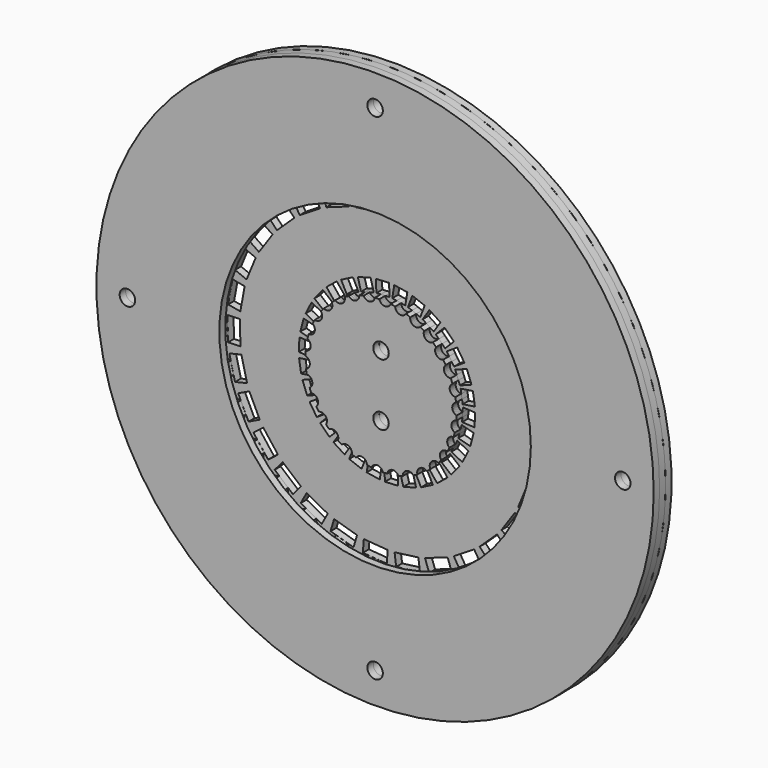
from build123d import *

# Parameters (mm, degrees)
F0_R     = 57.15
F0_R_2   = 1.5875
F1_DEPTH = 1.524
F2_R     = 57.15
F2_R_2   = 1.5875
F3_DEPTH = 1.524
F4_R     = 57.15
F4_R_2   = 1.5875
F4_R_3   = 31.9484375
F5_DEPTH = 1.524


# Not quite as in the source:
# - ends of sketch curves that miss each other by under 0.0002 mm in the source are joined


with BuildPart() as f1:
    # F0 (on Front) → F1 (new body)
    with BuildSketch(Plane.XZ):
        Circle(F0_R)
        with Locations((0, -50.8)):
            Circle(F0_R_2, mode=Mode.SUBTRACT)
        with Locations((-50.8, 0)):
            Circle(F0_R_2, mode=Mode.SUBTRACT)
        with BuildLine():
            Line((32.9977496, 2.3871936), (32.619442, 2.1111972))
            ThreePointArc((32.619442, 2.1111972), (32.6746635452, 0.9236684319), (32.6866413585, -0.2650997267))
            Line((32.6866413585, -0.2650997267), (33.0799349585, -0.5192013267))
            Line((33.0799349585, -0.5192013267), (33.414843, -0.841502))
            Line((33.414843, -0.841502), (33.6824574, -1.2215876))
            Line((33.6824574, -1.2215876), (33.8737448, -1.6489934))
            Line((33.8737448, -1.6489934), (33.979739, -2.1132038))
            Line((33.979739, -2.1132038), (33.99155, -2.6038048))
            Line((33.99155, -2.6038048), (33.9051392, -3.0867858))
            Line((33.9051392, -3.0867858), (33.7296506, -3.5295078))
            Line((33.7296506, -3.5295078), (33.475549, -3.9226998))
            Line((33.475549, -3.9226998), (33.1531468, -4.2575988))
            Line((33.1531468, -4.2575988), (32.7730612, -4.5251878))
            Line((32.7730612, -4.5251878), (32.3456554, -4.7165006))
            ThreePointArc((32.3456554, -4.7165006), (32.1527624461, -5.8895388824), (31.9173428687, -7.0547874079))
            Line((31.9173428687, -7.0547874079), (32.2491608, -7.3851008))
            Line((32.2491608, -7.3851008), (32.5097394, -7.7700886))
            Line((32.5097394, -7.7700886), (32.6924416, -8.1974944))
            Line((32.6924416, -8.1974944), (32.790638, -8.655304))
            Line((32.790638, -8.655304), (32.7979532, -9.1314016))
            Line((32.7979532, -9.1314016), (32.707453, -9.6136968))
            Line((32.707453, -9.6136968), (32.522541, -10.068306))
            Line((32.522541, -10.068306), (32.2588382, -10.4646984))
            Line((32.2588382, -10.4646984), (31.9285366, -10.7966002))
            Line((31.9285366, -10.7966002), (31.5436504, -11.0571026))
            Line((31.5436504, -11.0571026), (31.116143, -11.2398048))
            Line((31.116143, -11.2398048), (30.6583588, -11.3381028))
            ThreePointArc((30.6583588, -11.3381028), (30.2257804843, -12.4454407427), (29.7532339872, -13.5363166508))
            Line((29.7532339872, -13.5363166508), (30.008957, -13.9283948))
            Line((30.008957, -13.9283948), (30.1837598, -14.3591026))
            Line((30.1837598, -14.3591026), (30.2736504, -14.8151088))
            Line((30.2736504, -14.8151088), (30.2745394, -15.283307))
            Line((30.2745394, -15.283307), (30.1825406, -15.7504892))
            Line((30.1825406, -15.7504892), (29.9937424, -16.2034982))
            Line((29.9937424, -16.2034982), (29.7184572, -16.6095934))
            Line((29.7184572, -16.6095934), (29.378148, -16.9425874))
            Line((29.378148, -16.9425874), (28.9860482, -17.1984924))
            Line((28.9860482, -17.1984924), (28.5553404, -17.3733968))
            Line((28.5553404, -17.3733968), (28.0993596, -17.4631858))
            Line((28.0993596, -17.4631858), (27.6313593695, -17.4640997638))
            ThreePointArc((27.6313593695, -17.4640997638), (26.9779494763, -18.457438696), (26.2888462743, -19.4263574232))
            Line((26.2888462743, -19.4263574232), (26.4574528, -19.8629016))
            Line((26.4574528, -19.8629016), (26.538936, -20.320508))
            Line((26.538936, -20.320508), (26.5320526, -20.7853026))
            Line((26.5320526, -20.7853026), (26.435558, -21.2433916))
            Line((26.435558, -21.2433916), (26.2484362, -21.6812876))
            Line((26.2484362, -21.6812876), (25.9696458, -22.0850968))
            Line((25.9696458, -22.0850968), (25.6158492, -22.4251012))
            Line((25.6158492, -22.4251012), (25.2137418, -22.6800918))
            Line((25.2137418, -22.6800918), (24.776938, -22.8489002))
            Line((24.776938, -22.8489002), (24.319357, -22.9303072))
            Line((24.319357, -22.9303072), (23.854537, -22.9233984))
            Line((23.854537, -22.9233984), (23.3968997813, -22.8269989659))
            ThreePointArc((23.3968997813, -22.8269989659), (22.5511344494, -23.6629063348), (21.675524425, -24.4674976666))
            Line((21.675524425, -24.4674976666), (21.7497406, -24.9292872))
            Line((21.7497406, -24.9292872), (21.7342466, -25.3938024))
            Line((21.7342466, -25.3938024), (21.6308432, -25.8469892))
            Line((21.6308432, -25.8469892), (21.4412576, -26.2751062))
            Line((21.4412576, -26.2751062), (21.1672424, -26.6644882))
            Line((21.1672424, -26.6644882), (20.8105502, -27.0013938))
            Line((20.8105502, -27.0013938), (20.3937362, -27.2604992))
            Line((20.3937362, -27.2604992), (19.9474582, -27.426285))
            Line((19.9474582, -27.426285), (19.4850512, -27.5006054))
            Line((19.4850512, -27.5006054), (19.020536, -27.4851876))
            Line((19.020536, -27.4851876), (18.5673492, -27.3817842))
            Line((18.5673492, -27.3817842), (18.1398949027, -27.1924808373))
            ThreePointArc((18.1398949027, -27.1924808373), (17.1386971258, -27.8343647672), (16.1148119576, -28.43940289))
            Line((16.1148119576, -28.43940289), (16.0913572, -28.9061906))
            Line((16.0913572, -28.9061906), (15.979648, -29.3573962))
            Line((15.979648, -29.3573962), (15.7842458, -29.7791886))
            Line((15.7842458, -29.7791886), (15.5098496, -30.1584868))
            Line((15.5098496, -30.1584868), (15.1608536, -30.4824892))
            Line((15.1608536, -30.4824892), (14.7418552, -30.7379878))
            Line((14.7418552, -30.7379878), (14.2803372, -30.904688))
            Line((14.2803372, -30.904688), (13.8092434, -30.9740046))
            Line((13.8092434, -30.9740046), (13.3416548, -30.9505858))
            Line((13.3416548, -30.9505858), (12.8904492, -30.838902))
            Line((12.8904492, -30.838902), (12.4686568, -30.6434998))
            Line((12.4686568, -30.6434998), (12.0901433801, -30.3696433008))
            ThreePointArc((12.0901433801, -30.3696433008), (10.9771857627, -30.7894169139), (9.8496922142, -31.1684193447))
            Line((9.8496922142, -31.1684193447), (9.729851, -31.619698))
            Line((9.729851, -31.619698), (9.5267526, -32.0378074))
            Line((9.5267526, -32.0378074), (9.2479368, -32.4096888))
            Line((9.2479368, -32.4096888), (8.9006426, -32.723709))
            Line((8.9006426, -32.723709), (8.4919566, -32.9680062))
            Line((8.4919566, -32.9680062), (8.0290416, -33.1307948))
            Line((8.0290416, -33.1307948), (7.5429364, -33.1979016))
            Line((7.5429364, -33.1979016), (7.0676516, -33.1678026))
            Line((7.0676516, -33.1678026), (6.6151506, -33.0475844))
            Line((6.6151506, -33.0475844), (6.1970412, -32.844486))
            Line((6.1970412, -32.844486), (5.8250582, -32.5656956))
            Line((5.8250582, -32.5656956), (5.512130156, -32.2196092824))
            ThreePointArc((5.512130156, -32.2196092824), (4.3359328094, -32.3988655332), (3.1539910498, -32.5351985029))
            Line((3.1539910498, -32.5351985029), (2.9431488, -32.9511914))
            Line((2.9431488, -32.9511914), (2.6575512, -33.3178912))
            Line((2.6575512, -33.3178912), (2.3075392, -33.6237072))
            Line((2.3075392, -33.6237072), (1.90246, -33.8586064))
            Line((1.90246, -33.8586064), (1.4518386, -34.012505))
            Line((1.4518386, -34.012505), (0.9652508, -34.075497))
            Line((0.9652508, -34.075497), (0.4758436, -34.0400894))
            Line((0.4758436, -34.0400894), (0.0173482, -33.9118956))
            Line((0.0173482, -33.9118956), (-0.4003548, -33.7001866))
            Line((-0.4003548, -33.7001866), (-0.7671562, -33.4146906))
            Line((-0.7671562, -33.4146906), (-1.0729468, -33.064704))
            Line((-1.0729468, -33.064704), (-1.3067527256, -32.6615859762))
            ThreePointArc((-1.3067527256, -32.6615859762), (-2.4956293633, -32.5923094494), (-3.6811934951, -32.4797724071))
            Line((-3.6811934951, -32.4797724071), (-3.8585394, -32.7178924))
            Line((-3.8585394, -32.7178924), (-4.0768524, -32.943292))
            Line((-4.0768524, -32.943292), (-4.3233594, -33.1392022))
            Line((-4.3233594, -33.1392022), (-4.5954442, -33.302702))
            Line((-4.5954442, -33.302702), (-4.8905414, -33.4304894))
            Line((-4.8905414, -33.4304894), (-5.2000404, -33.518094))
            Line((-5.2000404, -33.518094), (-5.5141622, -33.5635854))
            Line((-5.5141622, -33.5635854), (-5.829046, -33.5677002))
            Line((-5.829046, -33.5677002), (-6.1406532, -33.531302))
            Line((-6.1406532, -33.531302), (-6.4448436, -33.4548988))
            Line((-6.4448436, -33.4548988), (-6.7377564, -33.339405))
            Line((-6.7377564, -33.339405), (-7.015353, -33.1855064))
            Line((-7.015353, -33.1855064), (-7.2736456, -32.9938888))
            Line((-7.2736456, -32.9938888), (-7.5042522, -32.7697846))
            Line((-7.5042522, -32.7697846), (-7.7007466, -32.520509))
            Line((-7.7007466, -32.520509), (-7.8618588, -32.249999))
            Line((-7.8618588, -32.249999), (-7.9860394, -31.9619884))
            Line((-7.9860394, -31.9619884), (-8.0674082753, -31.6765485002))
            ThreePointArc((-8.0674082753, -31.6765485002), (-9.2168478354, -31.3613857657), (-10.3540337201, -31.00452849))
            Line((-10.3540337201, -31.00452849), (-10.5767632, -31.2002932))
            Line((-10.5767632, -31.2002932), (-10.8370624, -31.3752992))
            Line((-10.8370624, -31.3752992), (-11.11885, -31.5156088))
            Line((-11.11885, -31.5156088), (-11.4190526, -31.618809))
            Line((-11.4190526, -31.618809), (-11.7342412, -31.6824868))
            Line((-11.7342412, -31.6824868), (-12.0551448, -31.703899))
            Line((-12.0551448, -31.703899), (-12.371959, -31.683198))
            Line((-12.371959, -31.683198), (-12.6807468, -31.6219078))
            Line((-12.6807468, -31.6219078), (-12.9779522, -31.5215016))
            Line((-12.9779522, -31.5215016), (-13.2596636, -31.3835034))
            Line((-13.2596636, -31.3835034), (-13.5221472, -31.2095896))
            Line((-13.5221472, -31.2095896), (-13.7616438, -31.0013858))
            Line((-13.7616438, -31.0013858), (-13.974445, -30.7601874))
            Line((-13.974445, -30.7601874), (-14.1534388, -30.4930048))
            Line((-14.1534388, -30.4930048), (-14.29385, -30.2082962))
            Line((-14.29385, -30.2082962), (-14.3951452, -29.9101002))
            Line((-14.3951452, -29.9101002), (-14.4567402, -29.6025062))
            Line((-14.4567402, -29.6025062), (-14.4769569648, -29.3070728358))
            ThreePointArc((-14.4769569648, -29.3070728358), (-15.5358976669, -28.7597406951), (-16.574177945, -28.1741623941))
            Line((-16.574177945, -28.1741623941), (-16.832453, -28.3192982))
            Line((-16.832453, -28.3192982), (-17.1234608, -28.4362906))
            Line((-17.1234608, -28.4362906), (-17.4283624, -28.5150052))
            Line((-17.4283624, -28.5150052), (-17.7434494, -28.5534862))
            Line((-17.7434494, -28.5534862), (-18.0650388, -28.5501842))
            Line((-18.0650388, -28.5501842), (-18.3833516, -28.5044896))
            Line((-18.3833516, -28.5044896), (-18.6888628, -28.418409))
            Line((-18.6888628, -28.418409), (-18.978245, -28.294203))
            Line((-18.978245, -28.294203), (-19.2480438, -28.1342084))
            Line((-19.2480438, -28.1342084), (-19.4948556, -27.9406858))
            Line((-19.4948556, -27.9406858), (-19.7154546, -27.7159974))
            Line((-19.7154546, -27.7159974), (-19.9064626, -27.4624038))
            Line((-19.9064626, -27.4624038), (-20.0644506, -27.182191))
            Line((-20.0644506, -27.182191), (-20.1839576, -26.8835886))
            Line((-20.1839576, -26.8835886), (-20.2621388, -26.5759946))
            Line((-20.2621388, -26.5759946), (-20.2992482, -26.2632952))
            Line((-20.2992482, -26.2632952), (-20.2955398, -25.9497068))
            Line((-20.2955398, -25.9497068), (-20.2538547168, -25.6567373272))
            ThreePointArc((-20.2538547168, -25.6567373272), (-21.1760973494, -24.9009980164), (-22.0701641601, -24.1121267231))
            Line((-22.0701641601, -24.1121267231), (-22.3524572, -24.2002056))
            Line((-22.3524572, -24.2002056), (-22.6614482, -24.254206))
            Line((-22.6614482, -24.254206), (-22.9760526, -24.267795))
            Line((-22.9760526, -24.267795), (-23.2922572, -24.240109))
            Line((-23.2922572, -24.240109), (-23.6061504, -24.170005))
            Line((-23.6061504, -24.170005), (-23.9079532, -24.0591086))
            Line((-23.9079532, -24.0591086), (-24.1889534, -23.911306))
            Line((-24.1889534, -23.911306), (-24.4461538, -23.7295944))
            Line((-24.4461538, -23.7295944), (-24.6767604, -23.5169964))
            Line((-24.6767604, -23.5169964), (-24.8780554, -23.2764076))
            Line((-24.8780554, -23.2764076), (-25.0470416, -23.0106982))
            Line((-25.0470416, -23.0106982), (-25.1811536, -22.7229924))
            Line((-25.1811536, -22.7229924), (-25.277445, -22.4161858))
            Line((-25.277445, -22.4161858), (-25.3322582, -22.0992954))
            Line((-25.3322582, -22.0992954), (-25.3446534, -21.7821002))
            Line((-25.3446534, -21.7821002), (-25.3159514, -21.4684864))
            Line((-25.3159514, -21.4684864), (-25.2471428, -21.1624926))
            Line((-25.2471428, -21.1624926), (-25.1456817839, -20.8849584339))
            ThreePointArc((-25.1456817839, -20.8849584339), (-25.8907055694, -19.9539010293), (-26.6012743407, -18.9962892328))
            Line((-26.6012743407, -18.9962892328), (-26.895552, -19.0236856))
            Line((-26.895552, -19.0236856), (-27.2089626, -19.0123064))
            Line((-27.2089626, -19.0123064), (-27.5194522, -18.9601856))
            Line((-27.5194522, -18.9601856), (-27.8229568, -18.8672978))
            Line((-27.8229568, -18.8672978), (-28.1154632, -18.7334906))
            Line((-28.1154632, -18.7334906), (-28.3876496, -18.562193))
            Line((-28.3876496, -18.562193), (-28.6317436, -18.3592978))
            Line((-28.6317436, -18.3592978), (-28.8455608, -18.128107))
            Line((-28.8455608, -18.128107), (-29.0269422, -17.872202))
            Line((-29.0269422, -17.872202), (-29.1737542, -17.5949864))
            Line((-29.1737542, -17.5949864), (-29.2838632, -17.2999908))
            Line((-29.2838632, -17.2999908), (-29.3552626, -16.990695))
            Line((-29.3552626, -16.990695), (-29.3855394, -16.6705026))
            Line((-29.3855394, -16.6705026), (-29.3733474, -16.349091))
            Line((-29.3733474, -16.349091), (-29.3196518, -16.03629))
            Line((-29.3196518, -16.03629), (-29.226256, -15.7355032))
            Line((-29.226256, -15.7355032), (-29.0953444, -15.4504898))
            Line((-29.0953444, -15.4504898), (-28.9385182487, -15.200294824))
            ThreePointArc((-28.9385182487, -15.200294824), (-29.4737245717, -14.1345803276), (-29.9697003394, -13.0500522119))
            Line((-29.9697003394, -13.0500522119), (-30.2628554, -13.0157982))
            Line((-30.2628554, -13.0157982), (-30.5670458, -12.939395))
            Line((-30.5670458, -12.939395), (-30.8599586, -12.8239012))
            Line((-30.8599586, -12.8239012), (-31.1375552, -12.669901))
            Line((-31.1375552, -12.669901), (-31.3957462, -12.4782072))
            Line((-31.3957462, -12.4782072), (-31.6264544, -12.254103))
            Line((-31.6264544, -12.254103), (-31.8229488, -12.004802))
            Line((-31.8229488, -12.004802), (-31.984061, -11.7341904))
            Line((-31.984061, -11.7341904), (-32.1082416, -11.4462052))
            Line((-32.1082416, -11.4462052), (-32.194246, -11.144504))
            Line((-32.194246, -11.144504), (-32.2406518, -10.8331))
            Line((-32.2406518, -10.8331), (-32.2461636, -10.5157016))
            Line((-32.2461636, -10.5157016), (-32.209359, -10.196195))
            Line((-32.209359, -10.196195), (-32.1305428, -9.8843846))
            Line((-32.1305428, -9.8843846), (-32.0129408, -9.5895922))
            Line((-32.0129408, -9.5895922), (-31.8591438, -9.3147896))
            Line((-31.8591438, -9.3147896), (-31.6718442, -9.0632026))
            Line((-31.6718442, -9.0632026), (-31.4665376445, -8.8512038634))
            ThreePointArc((-31.4665376445, -8.8512038634), (-31.7684907231, -7.6973890602), (-32.0281507731, -6.5333268109))
            Line((-32.0281507731, -6.5333268109), (-32.307657, -6.4389))
            Line((-32.307657, -6.4389), (-32.589343, -6.3010034))
            Line((-32.589343, -6.3010034), (-32.851852, -6.1270896))
            Line((-32.851852, -6.1270896), (-33.0913486, -5.9187842))
            Line((-33.0913486, -5.9187842), (-33.3041498, -5.6775858))
            Line((-33.3041498, -5.6775858), (-33.4831436, -5.4104032))
            Line((-33.4831436, -5.4104032), (-33.6236564, -5.1256946))
            Line((-33.6236564, -5.1256946), (-33.7249516, -4.8276002))
            Line((-33.7249516, -4.8276002), (-33.7865466, -4.5200062))
            Line((-33.7865466, -4.5200062), (-33.8079588, -4.2071036))
            Line((-33.8079588, -4.2071036), (-33.7886548, -3.892804))
            Line((-33.7886548, -3.892804), (-33.7279488, -3.5811968))
            Line((-33.7279488, -3.5811968), (-33.6255614, -3.2763968))
            Line((-33.6255614, -3.2763968), (-33.4836516, -2.987802))
            Line((-33.4836516, -2.987802), (-33.3072486, -2.7237944))
            Line((-33.3072486, -2.7237944), (-33.0996544, -2.4869902))
            Line((-33.0996544, -2.4869902), (-32.864044, -2.279904))
            Line((-32.864044, -2.279904), (-32.6192040783, -2.1152603773))
            ThreePointArc((-32.6192040783, -2.1152603773), (-32.6746598877, -0.9237978064), (-32.6866103591, 0.2688947737))
            Line((-32.6866103591, 0.2688947737), (-32.940244, 0.4193032))
            Line((-32.940244, 0.4193032), (-33.1871574, 0.6128004))
            Line((-33.1871574, 0.6128004), (-33.4077564, 0.8375142))
            Line((-33.4077564, 0.8375142), (-33.598739, 1.0911078))
            Line((-33.598739, 1.0911078), (-33.7567524, 1.3711936))
            Line((-33.7567524, 1.3711936), (-33.8762594, 1.669796))
            Line((-33.8762594, 1.669796), (-33.9544406, 1.9774154))
            Line((-33.9544406, 1.9774154), (-33.99155, 2.2901148))
            Line((-33.99155, 2.2901148), (-33.9878416, 2.6037032))
            Line((-33.9878416, 2.6037032), (-33.9436456, 2.9142944))
            Line((-33.9436456, 2.9142944), (-33.859343, 3.2176974))
            Line((-33.859343, 3.2176974), (-33.735264, 3.5097974))
            Line((-33.735264, 3.5097974), (-33.571561, 3.7867082))
            Line((-33.571561, 3.7867082), (-33.3727552, 4.0395144))
            Line((-33.3727552, 4.0395144), (-33.1454506, 4.261104))
            Line((-33.1454506, 4.261104), (-32.893254, 4.4494958))
            Line((-32.893254, 4.4494958), (-32.6198484, 4.6031912))
            Line((-32.6198484, 4.6031912), (-32.3461281326, 4.7132574714))
            ThreePointArc((-32.3461281326, 4.7132574714), (-32.1526477116, 5.8901652181), (-31.9163603631, 7.0592310017))
            Line((-31.9163603631, 7.0592310017), (-32.1332606, 7.259193))
            Line((-32.1332606, 7.259193), (-32.334454, 7.4998072))
            Line((-32.334454, 7.4998072), (-32.5035418, 7.765415))
            Line((-32.5035418, 7.765415), (-32.6376538, 8.0530954))
            Line((-32.6376538, 8.0530954), (-32.7339452, 8.3600036))
            Line((-32.7339452, 8.3600036), (-32.78886, 8.676894))
            Line((-32.78886, 8.676894), (-32.8012552, 8.9941146))
            Line((-32.8012552, 8.9941146), (-32.7725532, 9.307703))
            Line((-32.7725532, 9.307703), (-32.7037446, 9.6136968))
            Line((-32.7037446, 9.6136968), (-32.595947, 9.9083114))
            Line((-32.595947, 9.9083114), (-32.4504558, 10.1875082))
            Line((-32.4504558, 10.1875082), (-32.2683632, 10.4475026))
            Line((-32.2683632, 10.4475026), (-32.0507614, 10.6843068))
            Line((-32.0507614, 10.6843068), (-31.8037464, 10.8903008))
            Line((-31.8037464, 10.8903008), (-31.535243, 11.0596934))
            Line((-31.535243, 11.0596934), (-31.2493406, 11.1915956))
            Line((-31.2493406, 11.1915956), (-30.9498492, 11.2849914))
            Line((-30.9498492, 11.2849914), (-30.6592035748, 11.335785695))
            ThreePointArc((-30.6592035748, 11.335785695), (-30.2252803113, 12.4466554249), (-29.7511225316, 13.5409567341))
            Line((-29.7511225316, 13.5409567341), (-29.9218604, 13.7818114))
            Line((-29.9218604, 13.7818114), (-30.068647, 14.0590016))
            Line((-30.068647, 14.0590016), (-30.1788576, 14.3539972))
            Line((-30.1788576, 14.3539972), (-30.2501554, 14.663293))
            Line((-30.2501554, 14.663293), (-30.2805592, 14.9835108))
            Line((-30.2805592, 14.9835108), (-30.2683418, 15.304897))
            Line((-30.2683418, 15.304897), (-30.2145446, 15.617698))
            Line((-30.2145446, 15.617698), (-30.1212504, 15.9185102))
            Line((-30.1212504, 15.9185102), (-29.9903388, 16.2034982))
            Line((-29.9903388, 16.2034982), (-29.8237402, 16.4693092))
            Line((-29.8237402, 16.4693092), (-29.6233596, 16.7121078))
            Line((-29.6233596, 16.7121078), (-29.3910512, 16.9285158))
            Line((-29.3910512, 16.9285158), (-29.1289486, 17.114901))
            Line((-29.1289486, 17.114901), (-28.8445448, 17.265015))
            Line((-28.8445448, 17.265015), (-28.5467552, 17.3748954))
            Line((-28.5467552, 17.3748954), (-28.2396438, 17.4444914))
            Line((-28.2396438, 17.4444914), (-27.9273508, 17.4735998))
            Line((-27.9273508, 17.4735998), (-27.6321427962, 17.4628601797))
            ThreePointArc((-27.6321427962, 17.4628601797), (-26.9767730523, 18.4591580754), (-26.2854981559, 19.4308874698))
            Line((-26.2854981559, 19.4308874698), (-26.4025634, 19.7020942))
            Line((-26.4025634, 19.7020942), (-26.4885424, 20.0037954))
            Line((-26.4885424, 20.0037954), (-26.5349482, 20.3151994))
            Line((-26.5349482, 20.3151994), (-26.5403584, 20.6325978))
            Line((-26.5403584, 20.6325978), (-26.5035538, 20.9521044))
            Line((-26.5035538, 20.9521044), (-26.424763, 21.2639148))
            Line((-26.424763, 21.2639148), (-26.307161, 21.5588088))
            Line((-26.307161, 21.5588088), (-26.153364, 21.8335098))
            Line((-26.153364, 21.8335098), (-25.9659628, 22.0850968))
            Line((-25.9659628, 22.0850968), (-25.7477514, 22.3103948))
            Line((-25.7477514, 22.3103948), (-25.5012444, 22.506305))
            Line((-25.5012444, 22.506305), (-25.2291596, 22.6698048))
            Line((-25.2291596, 22.6698048), (-24.9340624, 22.7975922))
            Line((-24.9340624, 22.7975922), (-24.6245634, 22.8852984))
            Line((-24.6245634, 22.8852984), (-24.3104416, 22.9308152))
            Line((-24.3104416, 22.9308152), (-23.9955578, 22.9350062))
            Line((-23.9955578, 22.9350062), (-23.6840522, 22.898608))
            Line((-23.6840522, 22.898608), (-23.3972842996, 22.826604841))
            ThreePointArc((-23.3972842996, 22.826604841), (-22.5492259163, 23.664725051), (-21.6711652219, 24.4713587504))
            Line((-21.6711652219, 24.4713587504), (-21.7292428, 24.7612916))
            Line((-21.7292428, 24.7612916), (-21.750655, 25.0742958))
            Line((-21.750655, 25.0742958), (-21.731351, 25.3884938))
            Line((-21.731351, 25.3884938), (-21.670645, 25.700101))
            Line((-21.670645, 25.700101), (-21.568156, 26.004901))
            Line((-21.568156, 26.004901), (-21.4262462, 26.2934958))
            Line((-21.4262462, 26.2934958), (-21.2499448, 26.5575034))
            Line((-21.2499448, 26.5575034), (-21.0423506, 26.7943076))
            Line((-21.0423506, 26.7943076), (-20.8068418, 27.0013938))
            Line((-20.8068418, 27.0013938), (-20.5465426, 27.1763998))
            Line((-20.5465426, 27.1763998), (-20.2646534, 27.316811))
            Line((-20.2646534, 27.316811), (-19.9644508, 27.4201128))
            Line((-19.9644508, 27.4201128), (-19.6492622, 27.4837906))
            Line((-19.6492622, 27.4837906), (-19.3283586, 27.5052028))
            Line((-19.3283586, 27.5052028), (-19.0115444, 27.4845018))
            Line((-19.0115444, 27.4845018), (-18.7027566, 27.4232116))
            Line((-18.7027566, 27.4232116), (-18.4055512, 27.3228054))
            Line((-18.4055512, 27.3228054), (-18.1397297596, 27.1925910022))
            ThreePointArc((-18.1397297596, 27.1925910022), (-17.1360817184, 27.8359750055), (-16.1096400436, 28.4423328655))
            Line((-16.1096400436, 28.4423328655), (-16.10614, 28.7383982))
            Line((-16.10614, 28.7383982), (-16.0620456, 29.0489132))
            Line((-16.0620456, 29.0489132), (-15.977743, 29.3522908))
            Line((-15.977743, 29.3522908), (-15.853664, 29.6444924))
            Line((-15.853664, 29.6444924), (-15.6900626, 29.9215048))
            Line((-15.6900626, 29.9215048), (-15.4912568, 30.1742094))
            Line((-15.4912568, 30.1742094), (-15.2638506, 30.3956974))
            Line((-15.2638506, 30.3956974), (-15.011654, 30.5841146))
            Line((-15.011654, 30.5841146), (-14.7381468, 30.73781))
            Line((-14.7381468, 30.73781), (-14.447139, 30.8548024))
            Line((-14.447139, 30.8548024), (-14.1422628, 30.9335932))
            Line((-14.1422628, 30.9335932), (-13.8271504, 30.9722012))
            Line((-13.8271504, 30.9722012), (-13.505561, 30.9690008))
            Line((-13.505561, 30.9690008), (-13.1872482, 30.9232046))
            Line((-13.1872482, 30.9232046), (-12.8817624, 30.836997))
            Line((-12.8817624, 30.836997), (-12.5923548, 30.712791))
            Line((-12.5923548, 30.712791), (-12.322556, 30.5527964))
            Line((-12.322556, 30.5527964), (-12.0893442178, 30.3699614348))
            ThreePointArc((-12.0893442178, 30.3699614348), (-10.9740110348, 30.7905485981), (-9.844084736, 31.170190838))
            Line((-9.844084736, 31.170190838), (-9.7790508, 31.4593986))
            Line((-9.7790508, 31.4593986), (-9.6713548, 31.7540132))
            Line((-9.6713548, 31.7540132), (-9.5258636, 32.0333116))
            Line((-9.5258636, 32.0333116), (-9.3437456, 32.293306))
            Line((-9.3437456, 32.293306), (-9.1261438, 32.5301102))
            Line((-9.1261438, 32.5301102), (-8.8791542, 32.7361042))
            Line((-8.8791542, 32.7361042), (-8.6106508, 32.9054968))
            Line((-8.6106508, 32.9054968), (-8.3247484, 33.0372974))
            Line((-8.3247484, 33.0372974), (-8.025257, 33.1307948))
            Line((-8.025257, 33.1307948), (-7.7162406, 33.1847952))
            Line((-7.7162406, 33.1847952), (-7.4017632, 33.1984096))
            Line((-7.4017632, 33.1984096), (-7.0855586, 33.1705966))
            Line((-7.0855586, 33.1705966), (-6.77164, 33.1005942))
            Line((-6.77164, 33.1005942), (-6.469761, 32.9895962))
            Line((-6.469761, 32.9895962), (-6.1887608, 32.8417936))
            Line((-6.1887608, 32.8417936), (-5.9315604, 32.6601074))
            Line((-5.9315604, 32.6601074), (-5.7009538, 32.4475094))
            Line((-5.7009538, 32.4475094), (-5.5105249583, 32.2198838584))
            ThreePointArc((-5.5105249583, 32.2198838584), (-4.3323934404, 32.3993390094), (-3.1485034454, 32.535730009))
            Line((-3.1485034454, 32.535730009), (-3.0245558, 32.805497))
            Line((-3.0245558, 32.805497), (-2.8579572, 33.0712064))
            Line((-2.8579572, 33.0712064), (-2.6575512, 33.3141066))
            Line((-2.6575512, 33.3141066), (-2.4253444, 33.5305908))
            Line((-2.4253444, 33.5305908), (-2.1632418, 33.7170014))
            Line((-2.1632418, 33.7170014), (-1.8787618, 33.8670138))
            Line((-1.8787618, 33.8670138), (-1.5809468, 33.9768942))
            Line((-1.5809468, 33.9768942), (-1.2738608, 34.046414))
            Line((-1.2738608, 34.046414), (-0.9615424, 34.075497))
            Line((-0.9615424, 34.075497), (-0.6480556, 34.0640924))
            Line((-0.6480556, 34.0640924), (-0.337439, 34.011997))
            Line((-0.337439, 34.011997), (-0.0339598, 33.9191092))
            Line((-0.0339598, 33.9191092), (0.2585466, 33.785302))
            Line((0.2585466, 33.785302), (0.5307584, 33.614106))
            Line((0.5307584, 33.614106), (0.7747508, 33.4112108))
            Line((0.7747508, 33.4112108), (0.9885426, 33.1799946))
            Line((0.9885426, 33.1799946), (1.1699494, 32.9241912))
            Line((1.1699494, 32.9241912), (1.3090614558, 32.6614935248))
            ThreePointArc((1.3090614558, 32.6614935248), (2.4977560478, 32.592146537), (3.6831363001, 32.4795521545))
            Line((3.6831363001, 32.4795521545), (3.9757604, 32.8426064))
            Line((3.9757604, 32.8426064), (4.3313604, 33.1419962))
            Line((4.3313604, 33.1419962), (4.737354, 33.3683102))
            Line((4.737354, 33.3683102), (5.1824382, 33.513903))
            Line((5.1824382, 33.513903), (5.6551576, 33.570799))
            Line((5.6551576, 33.570799), (6.1443362, 33.531302))
            Line((6.1443362, 33.531302), (6.6157602, 33.394904))
            Line((6.6157602, 33.394904), (7.0375526, 33.1741018))
            Line((7.0375526, 33.1741018), (7.4020426, 32.8803))
            Line((7.4020426, 32.8803), (7.7014578, 32.5247))
            Line((7.7014578, 32.5247), (7.927848, 32.118808))
            Line((7.927848, 32.118808), (8.0730083687, 31.6751217368))
            ThreePointArc((8.0730083687, 31.6751217368), (9.2202072166, 31.3603982763), (10.3551947172, 31.0041407482))
            Line((10.3551947172, 31.0041407482), (10.7173522, 31.2986928))
            Line((10.7173522, 31.2986928), (11.1274606, 31.5176154))
            Line((11.1274606, 31.5176154), (11.5716558, 31.6545976))
            Line((11.5716558, 31.6545976), (12.0371362, 31.7045086))
            Line((12.0371362, 31.7045086), (12.5114558, 31.6619128))
            Line((12.5114558, 31.6619128), (12.9816606, 31.5216032))
            Line((12.9816606, 31.5216032), (13.4143496, 31.2902092))
            Line((13.4143496, 31.2902092), (13.781151, 30.9865014))
            Line((13.781151, 30.9865014), (14.076553, 30.6232052))
            Line((14.076553, 30.6232052), (14.2954502, 30.2131984))
            Line((14.2954502, 30.2131984), (14.4324578, 29.7690032))
            Line((14.4324578, 29.7690032), (14.4822399679, 29.3044625727))
            ThreePointArc((14.4822399679, 29.3044625727), (15.5387665805, 28.7581907345), (16.574720086, 28.1738434587))
            Line((16.574720086, 28.1738434587), (16.9906442, 28.386913))
            Line((16.9906442, 28.386913), (17.4372524, 28.5157926))
            Line((17.4372524, 28.5157926), (17.900142, 28.5573978))
            Line((17.900142, 28.5573978), (18.3659526, 28.5093156))
            Line((18.3659526, 28.5093156), (18.8209428, 28.369006))
            Line((18.8209428, 28.369006), (19.2517522, 28.1339036))
            Line((19.2517522, 28.1339036), (19.6268594, 27.8175974))
            Line((19.6268594, 27.8175974), (19.9224392, 27.4443952))
            Line((19.9224392, 27.4443952), (20.1359516, 27.0277082))
            Line((20.1359516, 27.0277082), (20.2648566, 26.5811))
            Line((20.2648566, 26.5811), (20.306538, 26.1181088))
            Line((20.306538, 26.1181088), (20.2585230706, 25.6530513617))
            ThreePointArc((20.2585230706, 25.6530513617), (21.1781930983, 24.8992156153), (22.0698353928, 24.1124276443))
            Line((22.0698353928, 24.1124276443), (22.5213418, 24.234394))
            Line((22.5213418, 24.234394), (22.9850442, 24.2675918))
            Line((22.9850442, 24.2675918), (23.4465368, 24.2121944))
            Line((23.4465368, 24.2121944), (23.8920528, 24.0683034))
            Line((23.8920528, 24.0683034), (24.308054, 23.836503))
            Line((24.308054, 23.836503), (24.6804434, 23.5169964))
            Line((24.6804434, 23.5169964), (24.9816366, 23.1295956))
            Line((24.9816366, 23.1295956), (25.1931424, 22.7030026))
            Line((25.1931424, 22.7030026), (25.3153418, 22.2510096))
            Line((25.3153418, 22.2510096), (25.3485396, 21.7874088))
            Line((25.3485396, 21.7874088), (25.2930406, 21.3258146))
            Line((25.2930406, 21.3258146), (25.1493352092, 20.8805588934))
            ThreePointArc((25.1493352092, 20.8805588934), (25.8920697512, 19.9521308428), (26.600548474, 18.9973056523))
            Line((26.600548474, 18.9973056523), (27.0678402, 19.0227966))
            Line((27.0678402, 19.0227966), (27.5282406, 18.9589156))
            Line((27.5282406, 18.9589156), (27.9681432, 18.8087))
            Line((27.9681432, 18.8087), (28.3740606, 18.5752994))
            Line((28.3740606, 18.5752994), (28.7326578, 18.262092))
            Line((28.7326578, 18.262092), (29.030549, 17.8721004))
            Line((29.030549, 17.8721004), (29.2446456, 17.430496))
            Line((29.2446456, 17.430496), (29.3628572, 16.9693082))
            Line((29.3628572, 16.9693082), (29.3884604, 16.5017958))
            Line((29.3884604, 16.5017958), (29.3244524, 16.0413954))
            Line((29.3244524, 16.0413954), (29.1742368, 15.6014928))
            Line((29.1742368, 15.6014928), (28.9409894793, 15.1955891338))
            ThreePointArc((28.9409894793, 15.1955891338), (29.2811854609, 14.5292456504), (29.606018374, 13.8553411074))
            Line((29.606018374, 13.8553411074), (35.0563935935, 16.1819569767))
            Line((35.0563935935, 16.1819569767), (37.383466959, 9.629400447))
            Line((37.383466959, 9.629400447), (31.6549937182, 8.1515749316))
            ThreePointArc((31.6549937182, 8.1515749316), (31.8514967635, 7.3463565861), (32.0275206969, 6.5364148563))
            Line((32.0275206969, 6.5364148563), (32.4650608, 6.3696088))
            Line((32.4650608, 6.3696088), (32.8596498, 6.1239146))
            Line((32.8596498, 6.1239146), (33.2004416, 5.80771))
            Line((33.2004416, 5.80771), (33.476438, 5.429504))
            Line((33.476438, 5.429504), (33.6766408, 4.9973992))
            Line((33.6766408, 4.9973992), (33.7901534, 4.5200062))
            Line((33.7901534, 4.5200062), (33.8061554, 4.0295068))
            Line((33.8061554, 4.0295068), (33.7264502, 3.5601148))
            Line((33.7264502, 3.5601148), (33.5596484, 3.1225998))
            Line((33.5596484, 3.1225998), (33.3139542, 2.7280108))
            Line((33.3139542, 2.7280108), (32.9977496, 2.3871936))
        make_face(mode=Mode.SUBTRACT)
        with Locations((50.8, 0)):
            Circle(F0_R_2, mode=Mode.SUBTRACT)
        with Locations((0, 50.8)):
            Circle(F0_R_2, mode=Mode.SUBTRACT)
    extrude(amount=-F1_DEPTH)

    # F4 (on face) → F5 (join)
    with BuildSketch(Plane.XZ):
        Circle(F4_R)
        with Locations((0, -50.8)):
            Circle(F4_R_2, mode=Mode.SUBTRACT)
        with Locations((-50.8, 0)):
            Circle(F4_R_2, mode=Mode.SUBTRACT)
        Circle(F4_R_3, mode=Mode.SUBTRACT)
        with Locations((50.8, 0)):
            Circle(F4_R_2, mode=Mode.SUBTRACT)
        with Locations((0, 50.8)):
            Circle(F4_R_2, mode=Mode.SUBTRACT)
    extrude(amount=F5_DEPTH)


with BuildPart() as f1b:
    # F0 (on Front) → F1, piece 2 (new body)
    with BuildSketch(Plane.XZ):
        with BuildLine():
            Line((15.355951, -1.2993878), (15.4622053838, -1.2809594684))
            ThreePointArc((15.4622053838, -1.2809594684), (15.4939184447, -0.8118766662), (15.5114040441, -0.3420483493))
            Line((15.5114040441, -0.3420483493), (15.40764, -0.3125978))
            Line((15.40764, -0.3125978), (15.2636474, -0.2505964))
            Line((15.2636474, -0.2505964), (15.128748, -0.1704848))
            Line((15.128748, -0.1704848), (15.0049484, -0.0733044))
            Line((15.0049484, -0.0733044), (14.8939504, 0.0402082))
            Line((14.8939504, 0.0402082), (14.797659, 0.16891))
            Line((14.797659, 0.16891), (14.7191476, 0.3092958))
            Line((14.7191476, 0.3092958), (14.6606514, 0.4567936))
            Line((14.6606514, 0.4567936), (14.622145, 0.6094984))
            Line((14.622145, 0.6094984), (14.603857, 0.765302))
            Line((14.603857, 0.765302), (14.6058382, 0.9220962))
            Line((14.6058382, 0.9220962), (14.6281394, 1.0780014))
            Line((14.6281394, 1.0780014), (14.6708368, 1.2308078))
            Line((14.6708368, 1.2308078), (14.7342606, 1.3786104))
            Line((14.7342606, 1.3786104), (14.8165566, 1.5167102))
            Line((14.8165566, 1.5167102), (14.9150578, 1.6411956))
            Line((14.9150578, 1.6411956), (15.028037, 1.7507966))
            Line((15.028037, 1.7507966), (15.1537416, 1.8444972))
            Line((15.1537416, 1.8444972), (15.290546, 1.9213068))
            Line((15.290546, 1.9213068), (15.3906915317, 1.9614450456))
            ThreePointArc((15.3906915317, 1.9614450456), (15.3242047505, 2.4268088629), (15.2436501955, 2.8899448453))
            Line((15.2436501955, 2.8899448453), (15.1360378, 2.8972002))
            Line((15.1360378, 2.8972002), (14.9822408, 2.9279088))
            Line((14.9822408, 2.9279088), (14.8336508, 2.9782008))
            Line((14.8336508, 2.9782008), (14.692249, 3.0475936))
            Line((14.692249, 3.0475936), (14.5601436, 3.135503))
            Line((14.5601436, 3.135503), (14.439138, 3.2413956))
            Line((14.439138, 3.2413956), (14.3332454, 3.3624012))
            Line((14.3332454, 3.3624012), (14.245336, 3.4945066))
            Line((14.245336, 3.4945066), (14.1759432, 3.6359084))
            Line((14.1759432, 3.6359084), (14.1256512, 3.7844984))
            Line((14.1256512, 3.7844984), (14.0949426, 3.9382954))
            Line((14.0949426, 3.9382954), (14.0843508, 4.0953944))
            Line((14.0843508, 4.0953944), (14.09446, 4.2538142))
            Line((14.09446, 4.2538142), (14.1257528, 4.4114974))
            Line((14.1257528, 4.4114974), (14.1775434, 4.5636942))
            Line((14.1775434, 4.5636942), (14.2480538, 4.7059088))
            Line((14.2480538, 4.7059088), (14.33576, 4.8366934))
            Line((14.33576, 4.8366934), (14.4392396, 4.9544986))
            Line((14.4392396, 4.9544986), (14.5570448, 5.0580036))
            Line((14.5570448, 5.0580036), (14.6466922318, 5.1181108975))
            ThreePointArc((14.6466922318, 5.1181108975), (14.4849079042, 5.5595049688), (14.3098251473, 5.9957949218))
            Line((14.3098251473, 5.9957949218), (14.2029434, 5.9805062))
            Line((14.2029434, 5.9805062), (14.0461492, 5.9786012))
            Line((14.0461492, 5.9786012), (13.8903456, 5.9969146))
            Line((13.8903456, 5.9969146), (13.7377424, 6.035294))
            Line((13.7377424, 6.035294), (13.5902446, 6.0938156))
            Line((13.5902446, 6.0938156), (13.4498588, 6.1723016))
            Line((13.4498588, 6.1723016), (13.3210554, 6.268593))
            Line((13.3210554, 6.268593), (13.2075428, 6.379591))
            Line((13.2075428, 6.379591), (13.1102608, 6.5033906))
            Line((13.1102608, 6.5033906), (13.0301492, 6.6383154))
            Line((13.0301492, 6.6383154), (12.9681478, 6.782308))
            Line((12.9681478, 6.782308), (12.9251456, 6.9337936))
            Line((12.9251456, 6.9337936), (12.9021586, 7.0908926))
            Line((12.9021586, 7.0908926), (12.8999488, 7.2517))
            Line((12.8999488, 7.2517), (12.918948, 7.4113136))
            Line((12.918948, 7.4113136), (12.9582418, 7.565009))
            Line((12.9582418, 7.565009), (13.0168396, 7.7111098))
            Line((13.0168396, 7.7111098), (13.0936492, 7.8479142))
            Line((13.0936492, 7.8479142), (13.1873498, 7.9735934))
            Line((13.1873498, 7.9735934), (13.2626868448, 8.0511980567))
            ThreePointArc((13.2626868448, 8.0511980567), (13.0126922989, 8.4492894154), (12.75075251, 8.8396245917))
            Line((12.75075251, 8.8396245917), (12.6491492, 8.8022938))
            Line((12.6491492, 8.8022938), (12.4962412, 8.7678006))
            Line((12.4962412, 8.7678006), (12.3400566, 8.7533988))
            Line((12.3400566, 8.7533988), (12.1827544, 8.7592916))
            Line((12.1827544, 8.7592916), (12.0262396, 8.7858092))
            Line((12.0262396, 8.7858092), (11.8726458, 8.8334088))
            Line((11.8726458, 8.8334088), (11.7266466, 8.9008966))
            Line((11.7266466, 8.9008966), (11.59256, 8.9859104))
            Line((11.59256, 8.9859104), (11.4717576, 9.0866976))
            Line((11.4717576, 9.0866976), (11.365357, 9.2020136))
            Line((11.365357, 9.2020136), (11.2747552, 9.3300042))
            Line((11.2747552, 9.3300042), (11.201146, 9.4691962))
            Line((11.201146, 9.4691962), (11.1459518, 9.6180148))
            Line((11.1459518, 9.6180148), (11.110341, 9.774809))
            Line((11.110341, 9.774809), (11.095736, 9.9349052))
            Line((11.095736, 9.9349052), (11.10234, 10.0935028))
            Line((11.10234, 10.0935028), (11.1292386, 10.2485952))
            Line((11.1292386, 10.2485952), (11.1758476, 10.3984044))
            Line((11.1758476, 10.3984044), (11.2414558, 10.5407968))
            Line((11.2414558, 10.5407968), (11.2990760247, 10.6325694674))
            ThreePointArc((11.2990760247, 10.6325694674), (10.97184887, 10.9699218259), (10.6345539944, 11.2972082317))
            Line((10.6345539944, 11.2972082317), (10.5427526, 11.2395))
            Line((10.5427526, 11.2395), (10.4002586, 11.1739934))
            Line((10.4002586, 11.1739934), (10.250551, 11.1273082))
            Line((10.250551, 11.1273082), (10.0954586, 11.1004096))
            Line((10.0954586, 11.1004096), (9.936861, 11.0938056))
            Line((9.936861, 11.0938056), (9.7767394, 11.1084106))
            Line((9.7767394, 11.1084106), (9.6198436, 11.1440976))
            Line((9.6198436, 11.1440976), (9.4710504, 11.1992918))
            Line((9.4710504, 11.1992918), (9.3318584, 11.272901))
            Line((9.3318584, 11.272901), (9.2038424, 11.3635028))
            Line((9.2038424, 11.3635028), (9.0886534, 11.4699034))
            Line((9.0886534, 11.4699034), (8.9877392, 11.5907058))
            Line((8.9877392, 11.5907058), (8.9027508, 11.7247924))
            Line((8.9027508, 11.7247924), (8.8352376, 11.8707916))
            Line((8.8352376, 11.8707916), (8.787638, 12.0244108))
            Line((8.787638, 12.0244108), (8.7611458, 12.1807986))
            Line((8.7611458, 12.1807986), (8.755253, 12.3382024))
            Line((8.755253, 12.3382024), (8.7697564, 12.4943108))
            Line((8.7697564, 12.4943108), (8.8042496, 12.647295))
            Line((8.8042496, 12.647295), (8.8416703392, 12.7493340259))
            ThreePointArc((8.8416703392, 12.7493340259), (8.4515218549, 13.0112424783), (8.0536208309, 13.2612157815))
            Line((8.0536208309, 13.2612157815), (7.9755492, 13.1854956))
            Line((7.9755492, 13.1854956), (7.8498446, 13.0916934))
            Line((7.8498446, 13.0916934), (7.7130402, 13.0150108))
            Line((7.7130402, 13.0150108), (7.5668378, 12.956413))
            Line((7.5668378, 12.956413), (7.4131424, 12.9169922))
            Line((7.4131424, 12.9169922), (7.2534526, 12.897993))
            Line((7.2534526, 12.897993), (7.0926452, 12.9002028))
            Line((7.0926452, 12.9002028), (6.9356478, 12.9232914))
            Line((6.9356478, 12.9232914), (6.7842384, 12.9662936))
            Line((6.7842384, 12.9662936), (6.6402458, 13.028295))
            Line((6.6402458, 13.028295), (6.5053464, 13.1084066))
            Line((6.5053464, 13.1084066), (6.3815468, 13.2056124))
            Line((6.3815468, 13.2056124), (6.2705488, 13.3190996))
            Line((6.2705488, 13.3190996), (6.1742574, 13.447903))
            Line((6.1742574, 13.447903), (6.095746, 13.5883142))
            Line((6.095746, 13.5883142), (6.0372498, 13.735812))
            Line((6.0372498, 13.735812), (5.9987434, 13.8884152))
            Line((5.9987434, 13.8884152), (5.9804554, 14.0441934))
            Line((5.9804554, 14.0441934), (5.9823604, 14.201013))
            Line((5.9823604, 14.201013), (5.9977905442, 14.308988821))
            ThreePointArc((5.9977905442, 14.308988821), (5.5617739365, 14.4840368396), (5.1206569175, 14.6458023073))
            Line((5.1206569175, 14.6458023073), (5.0598578, 14.5551144))
            Line((5.0598578, 14.5551144), (4.9563528, 14.4373092))
            Line((4.9563528, 14.4373092), (4.838446, 14.3338042))
            Line((4.838446, 14.3338042), (4.7077376, 14.246098))
            Line((4.7077376, 14.246098), (4.56565, 14.175613))
            Line((4.56565, 14.175613), (4.4134532, 14.123797))
            Line((4.4134532, 14.123797), (4.2557446, 14.0926058))
            Line((4.2557446, 14.0926058), (4.0972486, 14.0824966))
            Line((4.0972486, 14.0824966), (3.9401496, 14.0931138))
            Line((3.9401496, 14.0931138), (3.7863526, 14.123797))
            Line((3.7863526, 14.123797), (3.6377372, 14.1741144))
            Line((3.6377372, 14.1741144), (3.496437, 14.2435072))
            Line((3.496437, 14.2435072), (3.3642554, 14.3313912))
            Line((3.3642554, 14.3313912), (3.2432498, 14.4373092))
            Line((3.2432498, 14.4373092), (3.1373572, 14.5583148))
            Line((3.1373572, 14.5583148), (3.0494478, 14.6903948))
            Line((3.0494478, 14.6903948), (2.980055, 14.8317966))
            Line((2.980055, 14.8317966), (2.9297376, 14.9803104))
            Line((2.9297376, 14.9803104), (2.8990544, 15.1341074))
            Line((2.8990544, 15.1341074), (2.8916733377, 15.2433224003))
            ThreePointArc((2.8916733377, 15.2433224003), (2.4289256895, 15.3238693706), (1.9639519033, 15.3903718413))
            Line((1.9639519033, 15.3903718413), (1.923161, 15.2886156))
            Line((1.923161, 15.2886156), (1.8463514, 15.1519128))
            Line((1.8463514, 15.1519128), (1.7526508, 15.0261066))
            Line((1.7526508, 15.0261066), (1.6430498, 14.9132036))
            Line((1.6430498, 14.9132036), (1.5186406, 14.8146008))
            Line((1.5186406, 14.8146008), (1.3805408, 14.7323048))
            Line((1.3805408, 14.7323048), (1.2327382, 14.669008))
            Line((1.2327382, 14.669008), (1.0798556, 14.626209))
            Line((1.0798556, 14.626209), (0.9239504, 14.6039078))
            Line((0.9239504, 14.6039078), (0.7671562, 14.6020028))
            Line((0.7671562, 14.6020028), (0.6113526, 14.6202908))
            Line((0.6113526, 14.6202908), (0.4587494, 14.6586956))
            Line((0.4587494, 14.6586956), (0.3112516, 14.7171918))
            Line((0.3112516, 14.7171918), (0.1708404, 14.7957032))
            Line((0.1708404, 14.7957032), (0.042037, 14.8919946))
            Line((0.042037, 14.8919946), (-0.0714502, 15.0029926))
            Line((-0.0714502, 15.0029926), (-0.1687576, 15.1267922))
            Line((-0.1687576, 15.1267922), (-0.2488438, 15.2616916))
            Line((-0.2488438, 15.2616916), (-0.3108452, 15.4057096))
            Line((-0.3108452, 15.4057096), (-0.3408561198, 15.5114302886))
            ThreePointArc((-0.3408561198, 15.5114302886), (-0.8119712293, 15.4939134893), (-1.2823366494, 15.4620912301))
            Line((-1.2823366494, 15.4620912301), (-1.298956, 15.347315))
            Line((-1.298956, 15.347315), (-1.377061, 15.1266144))
            Line((-1.377061, 15.1266144), (-1.495044, 14.9264116))
            Line((-1.495044, 14.9264116), (-1.6489426, 14.752193))
            Line((-1.6489426, 14.752193), (-1.8347436, 14.6098006))
            Line((-1.8347436, 14.6098006), (-2.048256, 14.5044922))
            Line((-2.048256, 14.5044922), (-2.2855428, 14.4420082))
            Line((-2.2855428, 14.4420082), (-2.5305512, 14.4281144))
            Line((-2.5305512, 14.4281144), (-2.7661616, 14.4622012))
            Line((-2.7661616, 14.4622012), (-2.9868622, 14.5403062))
            Line((-2.9868622, 14.5403062), (-3.1870396, 14.6583908))
            Line((-3.1870396, 14.6583908), (-3.3611566, 14.8123148))
            Line((-3.3611566, 14.8123148), (-3.5036506, 14.9981158))
            Line((-3.5036506, 14.9981158), (-3.5550842175, 15.1023848679))
            ThreePointArc((-3.5550842175, 15.1023848679), (-4.0138981356, 14.9869701491), (-4.468979786, 14.8576200034))
            Line((-4.468979786, 14.8576200034), (-4.4613576, 14.7414996))
            Line((-4.4613576, 14.7414996), (-4.491863, 14.5093944))
            Line((-4.491863, 14.5093944), (-4.5657516, 14.2889986))
            Line((-4.5657516, 14.2889986), (-4.6800516, 14.086713))
            Line((-4.6800516, 14.086713), (-4.8321468, 13.9087098))
            Line((-4.8321468, 13.9087098), (-5.0191416, 13.7613136))
            Line((-5.0191416, 13.7613136), (-5.2381404, 13.6507982))
            Line((-5.2381404, 13.6507982), (-5.4749446, 13.5863076))
            Line((-5.4749446, 13.5863076), (-5.7125616, 13.570712))
            Line((-5.7125616, 13.570712), (-5.9446414, 13.601192))
            Line((-5.9446414, 13.601192), (-6.1650626, 13.675106))
            Line((-6.1650626, 13.675106), (-6.3673482, 13.789406))
            Line((-6.3673482, 13.789406), (-6.5453514, 13.9415012))
            Line((-6.5453514, 13.9415012), (-6.6175683049, 14.0331194758))
            ThreePointArc((-6.6175683049, 14.0331194758), (-7.0423329784, 13.8248399164), (-7.460550178, 13.6037069776))
            Line((-7.460550178, 13.6037069776), (-7.4288396, 13.4914132))
            Line((-7.4288396, 13.4914132), (-7.41045, 13.2580126))
            Line((-7.41045, 13.2580126), (-7.4368406, 13.0271012))
            Line((-7.4368406, 13.0271012), (-7.5065636, 12.8055116))
            Line((-7.5065636, 12.8055116), (-7.618349, 12.5996954))
            Line((-7.618349, 12.5996954), (-7.7705458, 12.4167138))
            Line((-7.7705458, 12.4167138), (-7.9618586, 12.2630946))
            Line((-7.9618586, 12.2630946), (-8.179943, 12.1508012))
            Line((-8.179943, 12.1508012), (-8.4091526, 12.0861074))
            Line((-8.4091526, 12.0861074), (-8.6425532, 12.0676924))
            Line((-8.6425532, 12.0676924), (-8.8734392, 12.0941084))
            Line((-8.8734392, 12.0941084), (-9.0951558, 12.1639076))
            Line((-9.0951558, 12.1639076), (-9.300845, 12.275693))
            Line((-9.300845, 12.275693), (-9.3907588357, 12.3504777633))
            ThreePointArc((-9.3907588357, 12.3504777633), (-9.7628572729, 12.058493702), (-10.1258826716, 11.7553031697))
            Line((-10.1258826716, 11.7553031697), (-10.071354, 11.6516912))
            Line((-10.071354, 11.6516912), (-10.0048568, 11.427206))
            Line((-10.0048568, 11.427206), (-9.9827588, 11.1959136))
            Line((-9.9827588, 11.1959136), (-10.0048568, 10.9644942))
            Line((-10.0048568, 10.9644942), (-10.071354, 10.740009))
            Line((-10.071354, 10.740009), (-10.1822504, 10.5292906))
            Line((-10.1822504, 10.5292906), (-10.3374444, 10.3392986))
            Line((-10.3374444, 10.3392986), (-10.5274618, 10.1841046))
            Line((-10.5274618, 10.1841046), (-10.7381548, 10.0732082))
            Line((-10.7381548, 10.0732082), (-10.96264, 10.006711))
            Line((-10.96264, 10.006711), (-11.1940594, 9.984613))
            Line((-11.1940594, 9.984613), (-11.4253518, 10.006711))
            Line((-11.4253518, 10.006711), (-11.6498624, 10.0732082))
            Line((-11.6498624, 10.0732082), (-11.7536296428, 10.1278251719))
            ThreePointArc((-11.7536296428, 10.1278251719), (-12.0568361455, 9.7649042316), (-12.3488410307, 9.3929110338))
            Line((-12.3488410307, 9.3929110338), (-12.2738388, 9.3028008))
            Line((-12.2738388, 9.3028008), (-12.162155, 9.09701))
            Line((-12.162155, 9.09701), (-12.0923558, 8.875395))
            Line((-12.0923558, 8.875395), (-12.0659398, 8.6444074))
            Line((-12.0659398, 8.6444074), (-12.0843548, 8.4110068))
            Line((-12.0843548, 8.4110068), (-12.148947, 8.1818988))
            Line((-12.148947, 8.1818988), (-12.261342, 7.9637128))
            Line((-12.261342, 7.9637128), (-12.4149612, 7.7724))
            Line((-12.4149612, 7.7724), (-12.5979428, 7.6201016))
            Line((-12.5979428, 7.6201016), (-12.8036574, 7.5083924))
            Line((-12.8036574, 7.5083924), (-13.0253486, 7.4385932))
            Line((-13.0253486, 7.4385932), (-13.25626, 7.4122026))
            Line((-13.25626, 7.4122026), (-13.4896606, 7.4305922))
            Line((-13.4896606, 7.4305922), (-13.6026328062, 7.4625085079))
            ThreePointArc((-13.6026328062, 7.4625085079), (-13.823740967, 7.0444899155), (-14.0320069369, 6.6199270248))
            Line((-14.0320069369, 6.6199270248), (-13.9397486, 6.5472056))
            Line((-13.9397486, 6.5472056), (-13.7876534, 6.3692024))
            Line((-13.7876534, 6.3692024), (-13.6733534, 6.1668914))
            Line((-13.6733534, 6.1668914), (-13.5994394, 5.9464956))
            Line((-13.5994394, 5.9464956), (-13.5689594, 5.7144158))
            Line((-13.5689594, 5.7144158), (-13.584555, 5.4767988))
            Line((-13.584555, 5.4767988), (-13.6490456, 5.2400962))
            Line((-13.6490456, 5.2400962), (-13.759561, 5.0209958))
            Line((-13.759561, 5.0209958), (-13.9069572, 4.834001))
            Line((-13.9069572, 4.834001), (-14.0849604, 4.6819058))
            Line((-14.0849604, 4.6819058), (-14.287246, 4.5676058))
            Line((-14.287246, 4.5676058), (-14.5076418, 4.4936918))
            Line((-14.5076418, 4.4936918), (-14.739747, 4.4632118))
            Line((-14.739747, 4.4632118), (-14.857039258, 4.470910084))
            ThreePointArc((-14.857039258, 4.470910084), (-14.9863855469, 4.0160802696), (-15.1018112805, 3.5575199983))
            Line((-15.1018112805, 3.5575199983), (-14.9963632, 3.5055048))
            Line((-14.9963632, 3.5055048), (-14.8105622, 3.3630108))
            Line((-14.8105622, 3.3630108), (-14.6566636, 3.1888938))
            Line((-14.6566636, 3.1888938), (-14.5385536, 2.988691))
            Line((-14.5385536, 2.988691), (-14.4604486, 2.7680158))
            Line((-14.4604486, 2.7680158), (-14.4263618, 2.5324054))
            Line((-14.4263618, 2.5324054), (-14.4402556, 2.287397))
            Line((-14.4402556, 2.287397), (-14.5027396, 2.0501102))
            Line((-14.5027396, 2.0501102), (-14.608048, 1.8365978))
            Line((-14.608048, 1.8365978), (-14.7504404, 1.6507968))
            Line((-14.7504404, 1.6507968), (-14.924659, 1.4968982))
            Line((-14.924659, 1.4968982), (-15.1248618, 1.3788136))
            Line((-15.1248618, 1.3788136), (-15.3455624, 1.3007086))
            Line((-15.3455624, 1.3007086), (-15.4633549, 1.2836525))
            Line((-15.4633549, 1.2836525), (-15.5128087, 0.3399028))
            Line((-15.5128087, 0.3399028), (-15.3974546, 0.3105912))
            Line((-15.3974546, 0.3105912), (-15.1860504, 0.209804))
            Line((-15.1860504, 0.209804), (-14.9993604, 0.071501))
            Line((-14.9993604, 0.071501), (-14.8422614, -0.0997966))
            Line((-14.8422614, -0.0997966), (-14.7199604, -0.2993898))
            Line((-14.7199604, -0.2993898), (-14.6375628, -0.5228082))
            Line((-14.6375628, -0.5228082), (-14.6002502, -0.765302))
            Line((-14.6002502, -0.765302), (-14.6120612, -1.0103866))
            Line((-14.6120612, -1.0103866), (-14.6705574, -1.2410948))
            Line((-14.6705574, -1.2410948), (-14.7713446, -1.4523974))
            Line((-14.7713446, -1.4523974), (-14.9096476, -1.639189))
            Line((-14.9096476, -1.639189), (-15.0809452, -1.796288))
            Line((-15.0809452, -1.796288), (-15.2805638, -1.918589))
            Line((-15.2805638, -1.918589), (-15.3909635432, -1.9593094965))
            ThreePointArc((-15.3909635432, -1.9593094965), (-15.3241148376, -2.4273765539), (-15.243034738, -2.8931893244))
            Line((-15.243034738, -2.8931893244), (-15.125446, -2.8977844))
            Line((-15.125446, -2.8977844), (-14.897862, -2.952496))
            Line((-14.897862, -2.952496), (-14.6863562, -3.0489906))
            Line((-14.6863562, -3.0489906), (-14.4971516, -3.18389))
            Line((-14.4971516, -3.18389), (-14.3360394, -3.353689))
            Line((-14.3360394, -3.353689), (-14.2089632, -3.5550856))
            Line((-14.2089632, -3.5550856), (-14.1220444, -3.7844984))
            Line((-14.1220444, -3.7844984), (-14.082649, -4.0265858))
            Line((-14.082649, -4.0265858), (-14.0919454, -4.2645076))
            Line((-14.0919454, -4.2645076), (-14.1465554, -4.4921932))
            Line((-14.1465554, -4.4921932), (-14.24305, -4.7035974))
            Line((-14.24305, -4.7035974), (-14.3779494, -4.8929036))
            Line((-14.3779494, -4.8929036), (-14.5477484, -5.0539904))
            Line((-14.5477484, -5.0539904), (-14.6471866402, -5.1166958106))
            ThreePointArc((-14.6471866402, -5.1166958106), (-14.4844395565, -5.5607250629), (-14.3082352789, -5.9995879603))
            Line((-14.3082352789, -5.9995879603), (-14.1924532, -5.9796934))
            Line((-14.1924532, -5.9796934), (-13.9583414, -5.9857894))
            Line((-13.9583414, -5.9857894), (-13.7315448, -6.0362084))
            Line((-13.7315448, -6.0362084), (-13.5183626, -6.1287914))
            Line((-13.5183626, -6.1287914), (-13.3254496, -6.2614048))
            Line((-13.3254496, -6.2614048), (-13.159359, -6.4319912))
            Line((-13.159359, -6.4319912), (-13.0265424, -6.63829))
            Line((-13.0265424, -6.63829), (-12.9376424, -6.8669916))
            Line((-12.9376424, -6.8669916), (-12.897358, -7.101586))
            Line((-12.897358, -7.101586), (-12.9033524, -7.3355962))
            Line((-12.9033524, -7.3355962), (-12.953746, -7.5624944))
            Line((-12.953746, -7.5624944), (-13.0463544, -7.775702))
            Line((-13.0463544, -7.775702), (-13.179044, -7.9685896))
            Line((-13.179044, -7.9685896), (-13.2631145048, -8.0504935329))
            ThreePointArc((-13.2631145048, -8.0504935329), (-13.011575791, -8.4510086928), (-12.7479463703, -8.8436709477))
            Line((-12.7479463703, -8.8436709477), (-12.6389638, -8.8001856))
            Line((-12.6389638, -8.8001856), (-12.4087636, -8.7574882))
            Line((-12.4087636, -8.7574882), (-12.1763536, -8.7595964))
            Line((-12.1763536, -8.7595964), (-11.948541, -8.8059006))
            Line((-11.948541, -8.8059006), (-11.73226, -8.8954864))
            Line((-11.73226, -8.8954864), (-11.5343432, -9.027795))
            Line((-11.5343432, -9.027795), (-11.361547, -9.2019882))
            Line((-11.361547, -9.2019882), (-11.227054, -9.4071948))
            Line((-11.227054, -9.4071948), (-11.1388398, -9.6283018))
            Line((-11.1388398, -9.6283018), (-11.0961424, -9.858502))
            Line((-11.0961424, -9.858502), (-11.0982506, -10.0908866))
            Line((-11.0982506, -10.0908866), (-11.1445548, -10.3185976))
            Line((-11.1445548, -10.3185976), (-11.2341406, -10.534904))
            Line((-11.2341406, -10.534904), (-11.2992881957, -10.6323439919))
            ThreePointArc((-11.2992881957, -10.6323439919), (-10.9699726583, -10.9717980463), (-10.6304638155, -11.3010570991))
            Line((-10.6304638155, -11.3010570991), (-10.5331514, -11.2359948))
            Line((-10.5331514, -11.2359948), (-10.316845, -11.146409))
            Line((-10.316845, -11.146409), (-10.0890578, -11.1001048))
            Line((-10.0890578, -11.1001048), (-9.8566478, -11.0979966))
            Line((-9.8566478, -11.0979966), (-9.6264476, -11.140694))
            Line((-9.6264476, -11.140694), (-9.4053406, -11.2289082))
            Line((-9.4053406, -11.2289082), (-9.2001594, -11.3634012))
            Line((-9.2001594, -11.3634012), (-9.0259408, -11.5361974))
            Line((-9.0259408, -11.5361974), (-8.8936576, -11.7340888))
            Line((-8.8936576, -11.7340888), (-8.8040464, -11.9503952))
            Line((-8.8040464, -11.9503952), (-8.7578438, -12.1782078))
            Line((-8.7578438, -12.1782078), (-8.755761, -12.4105924))
            Line((-8.755761, -12.4105924), (-8.7984584, -12.6407926))
            Line((-8.7984584, -12.6407926), (-8.8417329604, -12.7492905978))
            ThreePointArc((-8.8417329604, -12.7492905978), (-8.4488794295, -13.0129584983), (-8.0481689864, -13.2645251878))
            Line((-8.0481689864, -13.2645251878), (-7.9666592, -13.1807966))
            Line((-7.9666592, -13.1807966), (-7.7737462, -13.0482086))
            Line((-7.7737462, -13.0482086), (-7.560564, -12.9556002))
            Line((-7.560564, -12.9556002), (-7.333742, -12.9052066))
            Line((-7.333742, -12.9052066), (-7.0997572, -12.8990852))
            Line((-7.0997572, -12.8990852), (-6.8651628, -12.939395))
            Line((-6.8651628, -12.939395), (-6.6365628, -13.028295))
            Line((-6.6365628, -13.028295), (-6.4301624, -13.1610862))
            Line((-6.4301624, -13.1610862), (-6.2595506, -13.3272022))
            Line((-6.2595506, -13.3272022), (-6.1269626, -13.5200898))
            Line((-6.1269626, -13.5200898), (-6.0343542, -13.7332974))
            Line((-6.0343542, -13.7332974), (-5.9839606, -13.960094))
            Line((-5.9839606, -13.960094), (-5.9778392, -14.1942058))
            Line((-5.9778392, -14.1942058), (-5.9975774426, -14.3090781433))
            ThreePointArc((-5.9975774426, -14.3090781433), (-5.5585185545, -14.4852864649), (-5.1142913554, -14.6480263661))
            Line((-5.1142913554, -14.6480263661), (-5.0521616, -14.549501))
            Line((-5.0521616, -14.549501), (-4.8910494, -14.379702))
            Line((-4.8910494, -14.379702), (-4.7017432, -14.2448026))
            Line((-4.7017432, -14.2448026), (-4.490339, -14.148308))
            Line((-4.490339, -14.148308), (-4.2626534, -14.093698))
            Line((-4.2626534, -14.093698), (-4.024757, -14.0844016))
            Line((-4.024757, -14.0844016), (-3.7826442, -14.123797))
            Line((-3.7826442, -14.123797), (-3.5532568, -14.2106904))
            Line((-3.5532568, -14.2106904), (-3.3518602, -14.337792))
            Line((-3.3518602, -14.337792), (-3.1820612, -14.4989042))
            Line((-3.1820612, -14.4989042), (-3.0471618, -14.6881088))
            Line((-3.0471618, -14.6881088), (-2.9506418, -14.8995892))
            Line((-2.9506418, -14.8995892), (-2.8959556, -15.1271986))
            Line((-2.8959556, -15.1271986), (-2.8914158619, -15.2433712415))
            ThreePointArc((-2.8914158619, -15.2433712415), (-2.4252620619, -15.3244496287), (-1.9568527394, -15.3912760955))
            Line((-1.9568527394, -15.3912760955), (-1.9166586, -15.282291))
            Line((-1.9166586, -15.282291), (-1.7943576, -15.0826978))
            Line((-1.7943576, -15.0826978), (-1.6372586, -14.9114002))
            Line((-1.6372586, -14.9114002), (-1.4505432, -14.7730972))
            Line((-1.4505432, -14.7730972), (-1.239139, -14.6722846))
            Line((-1.239139, -14.6722846), (-1.0083546, -14.6137884))
            Line((-1.0083546, -14.6137884), (-0.7632446, -14.6020028))
            Line((-0.7632446, -14.6020028), (-0.5207508, -14.63929))
            Line((-0.5207508, -14.63929), (-0.2974594, -14.7216876))
            Line((-0.2974594, -14.7216876), (-0.0978408, -14.8439886))
            Line((-0.0978408, -14.8439886), (0.0734568, -15.0010876))
            Line((0.0734568, -15.0010876), (0.2117598, -15.187803))
            Line((0.2117598, -15.187803), (0.312547, -15.3992072))
            Line((0.312547, -15.3992072), (0.3410526923, -15.5114259677))
            ThreePointArc((0.3410526923, -15.5114259677), (0.8121651805, -15.4939033239), (1.2825278079, -15.4620753754))
            Line((1.2825278079, -15.4620753754), (1.3013436, -15.3539952))
            Line((1.3013436, -15.3539952), (1.3479526, -15.2042876))
            Line((1.3479526, -15.2042876), (1.4134592, -15.0617936))
            Line((1.4134592, -15.0617936), (1.4972538, -14.9284944))
            Line((1.4972538, -14.9284944), (1.5984474, -14.8061934))
            Line((1.5984474, -14.8061934), (1.7164558, -14.6969988))
            Line((1.7164558, -14.6969988), (1.84785, -14.6042888))
            Line((1.84785, -14.6042888), (1.988439, -14.530705))
            Line((1.988439, -14.530705), (2.1362416, -14.4763998))
            Line((2.1362416, -14.4763998), (2.2893528, -14.4419066))
            Line((2.2893528, -14.4419066), (2.4455374, -14.4275048))
            Line((2.4455374, -14.4275048), (2.6028396, -14.4333976))
            Line((2.6028396, -14.4333976), (2.7593544, -14.4598898))
            Line((2.7593544, -14.4598898), (2.9129482, -14.5074894))
            Line((2.9129482, -14.5074894), (3.0588458, -14.5750026))
            Line((3.0588458, -14.5750026), (3.1929578, -14.6598894))
            Line((3.1929578, -14.6598894), (3.3137602, -14.7608036))
            Line((3.3137602, -14.7608036), (3.4201608, -14.8760942))
            Line((3.4201608, -14.8760942), (3.5107372, -15.0040848))
            Line((3.5107372, -15.0040848), (3.5618669003, -15.1007866244))
            ThreePointArc((3.5618669003, -15.1007866244), (4.0173992569, -14.9860320199), (4.4692487014, -14.8575391144))
            Line((4.4692487014, -14.8575391144), (4.4651422, -14.7484084))
            Line((4.4651422, -14.7484084), (4.4796456, -14.5921984))
            Line((4.4796456, -14.5921984), (4.5141388, -14.4391888))
            Line((4.5141388, -14.4391888), (4.5683424, -14.2913862))
            Line((4.5683424, -14.2913862), (4.6420532, -14.1507972))
            Line((4.6420532, -14.1507972), (4.7347378, -14.019403))
            Line((4.7347378, -14.019403), (4.8439578, -13.9013946))
            Line((4.8439578, -13.9013946), (4.9662588, -13.8000994))
            Line((4.9662588, -13.8000994), (5.099558, -13.7164064))
            Line((5.099558, -13.7164064), (5.2419504, -13.6507982))
            Line((5.2419504, -13.6507982), (5.3917596, -13.6041892))
            Line((5.3917596, -13.6041892), (5.546852, -13.5772906))
            Line((5.546852, -13.5772906), (5.7054496, -13.5706866))
            Line((5.7054496, -13.5706866), (5.8655458, -13.5852916))
            Line((5.8655458, -13.5852916), (6.02234, -13.6209024))
            Line((6.02234, -13.6209024), (6.1711586, -13.6761982))
            Line((6.1711586, -13.6761982), (6.3103506, -13.7497058))
            Line((6.3103506, -13.7497058), (6.4383412, -13.8403076))
            Line((6.4383412, -13.8403076), (6.5535556, -13.9467082))
            Line((6.5535556, -13.9467082), (6.6233859882, -14.0303745689))
            ThreePointArc((6.6233859882, -14.0303745689), (7.0452559928, -13.8233505521), (7.4606627933, -13.6036452165))
            Line((7.4606627933, -13.6036452165), (7.4340466, -13.4980934))
            Line((7.4340466, -13.4980934), (7.4157586, -13.3422898))
            Line((7.4157586, -13.3422898), (7.4177398, -13.1854956))
            Line((7.4177398, -13.1854956), (7.440041, -13.0295904))
            Line((7.440041, -13.0295904), (7.4827384, -12.8768094))
            Line((7.4827384, -12.8768094), (7.5461368, -12.7290068))
            Line((7.5461368, -12.7290068), (7.6284582, -12.590907))
            Line((7.6284582, -12.590907), (7.7269594, -12.4663962))
            Line((7.7269594, -12.4663962), (7.8399386, -12.3567952))
            Line((7.8399386, -12.3567952), (7.9656432, -12.2630946))
            Line((7.9656432, -12.2630946), (8.102346, -12.186285))
            Line((8.102346, -12.186285), (8.2485484, -12.1276872))
            Line((8.2485484, -12.1276872), (8.4022438, -12.0882918))
            Line((8.4022438, -12.0882918), (8.561959, -12.0692926))
            Line((8.561959, -12.0692926), (8.722741, -12.071604))
            Line((8.722741, -12.071604), (8.8797384, -12.0946926))
            Line((8.8797384, -12.0946926), (9.0311478, -12.1376948))
            Line((9.0311478, -12.1376948), (9.175242, -12.1996962))
            Line((9.175242, -12.1996962), (9.3100398, -12.2798078))
            Line((9.3100398, -12.2798078), (9.3954863355, -12.3468817525))
            ThreePointArc((9.3954863355, -12.3468817525), (9.7651225261, -12.0566593442), (10.1257992671, -11.7553750129))
            Line((10.1257992671, -11.7553750129), (10.077958, -11.6578888))
            Line((10.077958, -11.6578888), (10.0276406, -11.5094004))
            Line((10.0276406, -11.5094004), (9.9969574, -11.3555018))
            Line((9.9969574, -11.3555018), (9.9863402, -11.1984028))
            Line((9.9863402, -11.1984028), (9.9964494, -11.0400084))
            Line((9.9964494, -11.0400084), (10.0276406, -10.8822998))
            Line((10.0276406, -10.8822998), (10.0794566, -10.730103))
            Line((10.0794566, -10.730103), (10.1500432, -10.5878884))
            Line((10.1500432, -10.5878884), (10.2377494, -10.4571038))
            Line((10.2377494, -10.4571038), (10.3412544, -10.3392986))
            Line((10.3412544, -10.3392986), (10.4590596, -10.2357936))
            Line((10.4590596, -10.2357936), (10.5897426, -10.1480874))
            Line((10.5897426, -10.1480874), (10.7319572, -10.0776024))
            Line((10.7319572, -10.0776024), (10.884154, -10.0257864))
            Line((10.884154, -10.0257864), (11.0419388, -9.9945952))
            Line((11.0419388, -9.9945952), (11.2003586, -9.984486))
            Line((11.2003586, -9.984486), (11.3574576, -9.9951032))
            Line((11.3574576, -9.9951032), (11.5112546, -10.0257864))
            Line((11.5112546, -10.0257864), (11.6598446, -10.0761038))
            Line((11.6598446, -10.0761038), (11.7570785311, -10.12382126))
            ThreePointArc((11.7570785311, -10.12382126), (12.0583512596, -9.7630332065), (12.3485568402, -9.3932846468))
            Line((12.3485568402, -9.3932846468), (12.2817382, -9.3081856))
            Line((12.2817382, -9.3081856), (12.201652, -9.1733878))
            Line((12.201652, -9.1733878), (12.1396506, -9.0292936))
            Line((12.1396506, -9.0292936), (12.0966484, -8.8778842))
            Line((12.0966484, -8.8778842), (12.0735598, -8.7208868))
            Line((12.0735598, -8.7208868), (12.0712484, -8.5601048))
            Line((12.0712484, -8.5601048), (12.0902476, -8.4003896))
            Line((12.0902476, -8.4003896), (12.129643, -8.2466942))
            Line((12.129643, -8.2466942), (12.1882408, -8.1004918))
            Line((12.1882408, -8.1004918), (12.2649488, -7.9636874))
            Line((12.2649488, -7.9636874), (12.358751, -7.8380082))
            Line((12.358751, -7.8380082), (12.468352, -7.7250036))
            Line((12.468352, -7.7250036), (12.5928374, -7.6265024))
            Line((12.5928374, -7.6265024), (12.7309372, -7.5442064))
            Line((12.7309372, -7.5442064), (12.8787398, -7.480808))
            Line((12.8787398, -7.480808), (13.0315462, -7.4380852))
            Line((13.0315462, -7.4380852), (13.1874514, -7.4158094))
            Line((13.1874514, -7.4158094), (13.3442456, -7.4138028))
            Line((13.3442456, -7.4138028), (13.4999476, -7.4320908))
            Line((13.4999476, -7.4320908), (13.6048126034, -7.4585338048))
            ThreePointArc((13.6048126034, -7.4585338048), (13.8245284038, -7.0429444768), (14.0315528299, -6.6208894927))
            Line((14.0315528299, -6.6208894927), (13.9486386, -6.5517014))
            Line((13.9486386, -6.5517014), (13.842238, -6.436487))
            Line((13.842238, -6.436487), (13.7516362, -6.3083948))
            Line((13.7516362, -6.3083948), (13.6780524, -6.1692028))
            Line((13.6780524, -6.1692028), (13.6228582, -6.0203842))
            Line((13.6228582, -6.0203842), (13.5872474, -5.86359))
            Line((13.5872474, -5.86359), (13.5726424, -5.7034938))
            Line((13.5726424, -5.7034938), (13.5791448, -5.5448962))
            Line((13.5791448, -5.5448962), (13.606145, -5.3898038))
            Line((13.606145, -5.3898038), (13.652754, -5.2399946))
            Line((13.652754, -5.2399946), (13.7182606, -5.0976022))
            Line((13.7182606, -5.0976022), (13.8020552, -4.964303))
            Line((13.8020552, -4.964303), (13.9033504, -4.842002))
            Line((13.9033504, -4.842002), (14.0213588, -4.7328074))
            Line((14.0213588, -4.7328074), (14.152753, -4.6400974))
            Line((14.152753, -4.6400974), (14.293342, -4.5664882))
            Line((14.293342, -4.5664882), (14.4411446, -4.5122084))
            Line((14.4411446, -4.5122084), (14.5941542, -4.4776898))
            Line((14.5941542, -4.4776898), (14.7503388, -4.463288))
            Line((14.7503388, -4.463288), (14.8581122966, -4.4673427755))
            ThreePointArc((14.8581122966, -4.4673427755), (14.9866384112, -4.0151365633), (15.1014050573, -3.5592439911))
            Line((15.1014050573, -3.5592439911), (15.0060406, -3.5089084))
            Line((15.0060406, -3.5089084), (14.87805, -3.4183066))
            Line((14.87805, -3.4183066), (14.7627594, -3.311906))
            Line((14.7627594, -3.311906), (14.6618452, -3.191002))
            Line((14.6618452, -3.191002), (14.5768568, -3.0569916))
            Line((14.5768568, -3.0569916), (14.5094452, -2.9109924))
            Line((14.5094452, -2.9109924), (14.4618456, -2.7573986))
            Line((14.4618456, -2.7573986), (14.4353534, -2.6009092))
            Line((14.4353534, -2.6009092), (14.429359, -2.443607))
            Line((14.429359, -2.443607), (14.443837, -2.287397))
            Line((14.443837, -2.287397), (14.4783556, -2.1343874))
            Line((14.4783556, -2.1343874), (14.5325592, -1.9865848))
            Line((14.5325592, -1.9865848), (14.6062446, -1.8459958))
            Line((14.6062446, -1.8459958), (14.6989546, -1.7146016))
            Line((14.6989546, -1.7146016), (14.8081492, -1.5965932))
            Line((14.8081492, -1.5965932), (14.9304502, -1.4953996))
            Line((14.9304502, -1.4953996), (15.0637494, -1.411605))
            Line((15.0637494, -1.411605), (15.2061418, -1.3460984))
            Line((15.2061418, -1.3460984), (15.355951, -1.2993878))
        make_face()
        with Locations((0, -6.35)):
            Circle(F0_R_2, mode=Mode.SUBTRACT)
        with Locations((0, 6.35)):
            Circle(F0_R_2, mode=Mode.SUBTRACT)
    extrude(amount=-F1_DEPTH)


with BuildPart() as f3:
    # F2 (on face) → F3 (new body)
    with BuildSketch(Plane(origin=(0, 1.524, 0), x_dir=(-1, 0, 0), z_dir=(0, 1, 0))):
        Circle(F2_R)
        Polygon((-8.6523330286, -31.5951888649), (-13.2841238345, -29.9441293111), (-12.4312732657, -27.5515896756), (-7.7994824598, -29.2026492295), align=None, mode=Mode.SUBTRACT)
        Polygon((-1.894249654, -32.7036793725), (-6.7680993014, -32.0517028892), (-6.4313225248, -29.5341283813), (-1.5574728774, -30.1861048646), align=None, mode=Mode.SUBTRACT)
        Polygon((-29.2693419608, -14.7113713647), (-31.1416385873, -10.1645055142), (-28.7929667192, -9.1973755043), (-26.9206700927, -13.7442413548), align=None, mode=Mode.SUBTRACT)
        Polygon((-31.6884027087, -8.3044542277), (-32.5744385948, -3.4676759479), (-30.0760132066, -3.0099963883), (-29.1899773204, -7.8467746682), align=None, mode=Mode.SUBTRACT)
        Polygon((-20.7552205925, -25.3444203801), (-24.3150256236, -21.9521833806), (-22.5627743207, -20.1133752417), (-19.0029692896, -23.5056122413), align=None, mode=Mode.SUBTRACT)
        Polygon((-15.0322679313, -29.1058369935), (-19.2195684117, -26.5278535942), (-17.8879177131, -24.3649142939), (-13.7006172327, -26.9428976931), align=None, mode=Mode.SUBTRACT)
        Polygon((-25.5710705193, -20.4753309801), (-28.3477995393, -16.4170974149), (-26.2515294222, -14.9827851768), (-23.4748004023, -19.041018742), align=None, mode=Mode.SUBTRACT)
        Polygon((-5.8296039505, -14.435761638), (-6.9836883132, -16.6984346775), (-9.3997930023, -15.4660919609), (-8.2457086396, -13.2034189214), (-7.4537730758, -13.6073484483), (-6.6215395143, -14.0318321111), align=None, mode=Mode.SUBTRACT)
        Polygon((-2.700849507, -15.3323484251), (-3.35927818, -17.7855242612), (-5.9788036427, -17.0824476007), (-5.3203749697, -14.6292717647), (-4.461763427, -14.8597218002), (-3.5594610496, -15.1018983896), align=None, mode=Mode.SUBTRACT)
        Polygon((0.5459450201, -15.5588380133), (0.4119485292, -18.0953010902), (-2.2965118744, -17.9522183097), (-2.1625153836, -15.4157552328), (-1.2747533066, -15.4626540046), (-0.3418170568, -15.5119392415), align=None, mode=Mode.SUBTRACT)
        Polygon((-13.2013764629, -8.2522212631), (-15.4650161686, -9.4044084365), (-16.6953330477, -6.9872715315), (-14.4316933419, -5.8350843582), (-14.0284278312, -6.6273582552), (-13.6046419735, -7.4599473661), align=None, mode=Mode.SUBTRACT)
        Polygon((-14.6286279893, -5.3271699277), (-17.0823549198, -5.9835418883), (-17.7832354024, -3.3634279615), (-15.3295084719, -2.7070560009), (-15.0997782857, -3.5658604266), (-14.8583581756, -4.4683655021), align=None, mode=Mode.SUBTRACT)
        Polygon((-15.5573505225, 0.5392836934), (-15.5111959723, -0.3485173865), (-15.462692827, -1.281494624), (-15.4165382768, -2.1692957039), (-17.9531127908, -2.3011658474), (-18.0939250366, 0.4074135499), align=None, mode=Mode.SUBTRACT)
        Polygon((-8.7035767278, -12.9082627969), (-10.3028777557, -14.8815433705), (-12.4099663026, -13.1737938878), (-10.8106652747, -11.2005133142), (-10.1200170739, -11.7602686739), (-9.3942249286, -12.3485074371), align=None, mode=Mode.SUBTRACT)
        Polygon((-11.1971614377, -10.8166109308), (-13.1717820015, -12.4142572086), (-14.8777645257, -10.305737807), (-12.903143962, -8.7080915291), (-12.3439677647, -9.3992087264), (-11.756337635, -10.1254937334), align=None, mode=Mode.SUBTRACT)
        with Locations((0, -50.8)):
            Circle(F2_R_2, mode=Mode.SUBTRACT)
        Polygon((4.94662152, -32.3828621617), (0.0437236481, -32.7584632498), (-0.1502921286, -30.2258839562), (4.7526057434, -29.8502828681), align=None, mode=Mode.SUBTRACT)
        Polygon((11.5713015971, -30.6467584843), (6.8536356643, -32.033521574), (6.1373067548, -29.5966233624), (10.8549726876, -28.2098602728), align=None, mode=Mode.SUBTRACT)
        Polygon((3.76887913, -15.1053317207), (4.165171111, -17.6142264307), (1.4861484827, -18.0373909343), (1.0898565017, -15.5284962243), (1.9679696502, -15.389794031), (2.8907659815, -15.2440339141), align=None, mode=Mode.SUBTRACT)
        Polygon((6.8270951369, -13.9916499485), (7.7363557285, -16.3633255537), (5.2038570198, -17.334243022), (4.2945964281, -14.9625674168), (5.12468289, -14.6443262097), (5.9970086751, -14.3098911556), align=None, mode=Mode.SUBTRACT)
        Polygon((17.6902602691, -27.5712444017), (13.3640109147, -29.9085612914), (12.156675883, -27.6738483073), (16.4829252375, -25.3365314176), align=None, mode=Mode.SUBTRACT)
        Polygon((23.0360696801, -23.2907346372), (19.2903147604, -26.4764533632), (17.6447399408, -24.5415932873), (21.3904948606, -21.3558745613), align=None, mode=Mode.SUBTRACT)
        Polygon((27.3750923068, -17.9923080077), (24.3735392859, -21.8871973749), (22.3616441944, -20.336752877), (25.3631972153, -16.4418635098), align=None, mode=Mode.SUBTRACT)
        Polygon((9.5869343263, -12.2664659341), (10.9694244776, -14.3972688301), (8.6941320342, -15.8735055108), (7.3116418829, -13.7427026148), (8.0574228965, -13.2588310618), (8.8411533127, -12.7503374871), align=None, mode=Mode.SUBTRACT)
        Polygon((11.9277784824, -10.0051784974), (13.7230767398, -11.8019823729), (11.8044317597, -13.7190196392), (10.0091335022, -11.9222157637), (10.6380148586, -11.2938613736), (11.298897126, -10.6335328875), align=None, mode=Mode.SUBTRACT)
        Polygon((13.7473214829, -7.3066167502), (15.8769646979, -8.6908926537), (14.3988211733, -10.9649467782), (12.2691779584, -9.5806708746), (12.7536745246, -8.8352957494), (13.2628249167, -8.0519918754), align=None, mode=Mode.SUBTRACT)
        with Locations((0, -6.35)):
            Circle(F2_R_2, mode=Mode.SUBTRACT)
        Polygon((30.5176920393, -11.9075311816), (28.3915231873, -16.3413658349), (26.1012372937, -15.2430987794), (28.2274061456, -10.8092641261), align=None, mode=Mode.SUBTRACT)
        Polygon((14.9660405677, -4.28872079), (17.3369531125, -5.1999692221), (16.3639130084, -7.7316531273), (13.9930004637, -6.8204046952), (14.3119374149, -5.9905853045), (14.6471036165, -5.1185401806), align=None, mode=Mode.SUBTRACT)
        Polygon((15.5306718647, -1.0833871516), (18.0392334842, -1.4817821832), (17.6138233223, -4.1604491342), (15.1052617028, -3.7620541026), (15.2446999639, -2.8840575358), (15.3912336036, -1.9613837185), align=None, mode=Mode.SUBTRACT)
        Polygon((32.3265221896, -5.3023381042), (31.1686612879, -10.0813381934), (28.7000810755, -9.4832481207), (29.8579419773, -4.7042480315), align=None, mode=Mode.SUBTRACT)
        Polygon((32.7225282004, 1.5345925918), (32.5835793263, -3.3807076972), (30.0445935961, -3.3089340134), (30.1835424702, 1.6063662755), align=None, mode=Mode.SUBTRACT)
        with Locations((-50.8, 0)):
            Circle(F2_R_2, mode=Mode.SUBTRACT)
        Polygon((-32.7225282004, -1.5345925918), (-32.5835793263, 3.3807076972), (-30.0445935961, 3.3089340134), (-30.1835424702, -1.6063662755), align=None, mode=Mode.SUBTRACT)
        Polygon((-32.3265221896, 5.3023381042), (-31.1686612879, 10.0813381934), (-28.7000810755, 9.4832481207), (-29.8579419773, 4.7042480315), align=None, mode=Mode.SUBTRACT)
        Polygon((-15.5306718647, 1.0833871516), (-18.0392334842, 1.4817821832), (-17.6138233223, 4.1604491342), (-15.1052617028, 3.7620541026), (-15.2446999639, 2.8840575358), (-15.3912336036, 1.9613837185), align=None, mode=Mode.SUBTRACT)
        Polygon((-14.9660405677, 4.28872079), (-17.3369531125, 5.1999692221), (-16.3639130084, 7.7316531273), (-13.9930004637, 6.8204046952), (-14.3119374149, 5.9905853045), (-14.6471036165, 5.1185401806), align=None, mode=Mode.SUBTRACT)
        Polygon((-30.5176920393, 11.9075311816), (-28.3915231873, 16.3413658349), (-26.1012372937, 15.2430987794), (-28.2274061456, 10.8092641261), align=None, mode=Mode.SUBTRACT)
        Polygon((-13.7473214829, 7.3066167502), (-15.8769646979, 8.6908926537), (-14.3988211733, 10.9649467782), (-12.2691779584, 9.5806708746), (-12.7536745246, 8.8352957494), (-13.2628249167, 8.0519918754), align=None, mode=Mode.SUBTRACT)
        Polygon((-11.9277784824, 10.0051784974), (-13.7230767398, 11.8019823729), (-11.8044317597, 13.7190196392), (-10.0091335022, 11.9222157637), (-10.6380148586, 11.2938613736), (-11.298897126, 10.6335328875), align=None, mode=Mode.SUBTRACT)
        Polygon((-9.5869343263, 12.2664659341), (-10.9694244776, 14.3972688301), (-8.6941320342, 15.8735055108), (-7.3116418829, 13.7427026148), (-8.0574228965, 13.2588310618), (-8.8411533127, 12.7503374871), align=None, mode=Mode.SUBTRACT)
        Polygon((-27.3750923068, 17.9923080077), (-24.3735392859, 21.8871973749), (-22.3616441944, 20.336752877), (-25.3631972153, 16.4418635098), align=None, mode=Mode.SUBTRACT)
        Polygon((-23.0360696801, 23.2907346372), (-19.2903147604, 26.4764533632), (-17.6447399408, 24.5415932873), (-21.3904948606, 21.3558745613), align=None, mode=Mode.SUBTRACT)
        Polygon((-17.6902602691, 27.5712444017), (-13.3640109147, 29.9085612914), (-12.156675883, 27.6738483073), (-16.4829252375, 25.3365314176), align=None, mode=Mode.SUBTRACT)
        Polygon((-6.8270951369, 13.9916499485), (-7.7363557285, 16.3633255537), (-5.2038570198, 17.334243022), (-4.2945964281, 14.9625674168), (-5.12468289, 14.6443262097), (-5.9970086751, 14.3098911556), align=None, mode=Mode.SUBTRACT)
        Polygon((-3.76887913, 15.1053317207), (-4.165171111, 17.6142264307), (-1.4861484827, 18.0373909343), (-1.0898565017, 15.5284962243), (-1.9679696502, 15.389794031), (-2.8907659815, 15.2440339141), align=None, mode=Mode.SUBTRACT)
        Polygon((-11.5713015971, 30.6467584843), (-6.8536356643, 32.033521574), (-6.1373067548, 29.5966233624), (-10.8549726876, 28.2098602728), align=None, mode=Mode.SUBTRACT)
        Polygon((-4.94662152, 32.3828621617), (-0.0437236481, 32.7584632498), (0.1502921286, 30.2258839562), (-4.7526057434, 29.8502828681), align=None, mode=Mode.SUBTRACT)
        with Locations((0, 6.35)):
            Circle(F2_R_2, mode=Mode.SUBTRACT)
        Polygon((11.1971614377, 10.8166109308), (13.1717820015, 12.4142572086), (14.8777645257, 10.305737807), (12.903143962, 8.7080915291), (12.3439677647, 9.3992087264), (11.756337635, 10.1254937334), align=None, mode=Mode.SUBTRACT)
        Polygon((8.7035767278, 12.9082627969), (10.3028777557, 14.8815433705), (12.4099663026, 13.1737938878), (10.8106652747, 11.2005133142), (10.1200170739, 11.7602686739), (9.3942249286, 12.3485074371), align=None, mode=Mode.SUBTRACT)
        Polygon((15.4165382768, 2.1692957039), (17.9531127908, 2.3011658474), (18.0939250366, -0.4074135499), (15.5573505225, -0.5392836934), (15.5111959723, 0.3485173865), (15.462692827, 1.281494624), align=None, mode=Mode.SUBTRACT)
        Polygon((14.6286279893, 5.3271699277), (17.0823549198, 5.9835418883), (17.7832354024, 3.3634279615), (15.3295084719, 2.7070560009), (15.0997782857, 3.5658604266), (14.8583581756, 4.4683655021), align=None, mode=Mode.SUBTRACT)
        Polygon((13.2013764629, 8.2522212631), (15.4650161686, 9.4044084365), (16.6953330477, 6.9872715315), (14.4316933419, 5.8350843582), (14.0284278312, 6.6273582552), (13.6046419735, 7.4599473661), align=None, mode=Mode.SUBTRACT)
        Polygon((-0.5459450201, 15.5588380133), (-0.4119485292, 18.0953010902), (2.2965118744, 17.9522183097), (2.1625153836, 15.4157552328), (1.2747533066, 15.4626540046), (0.3418170568, 15.5119392415), align=None, mode=Mode.SUBTRACT)
        Polygon((2.700849507, 15.3323484251), (3.35927818, 17.7855242612), (5.9788036427, 17.0824476007), (5.3203749697, 14.6292717647), (4.461763427, 14.8597218002), (3.5594610496, 15.1018983896), align=None, mode=Mode.SUBTRACT)
        Polygon((5.8296039505, 14.435761638), (6.9836883132, 16.6984346775), (9.3997930023, 15.4660919609), (8.2457086396, 13.2034189214), (7.4537730758, 13.6073484483), (6.6215395143, 14.0318321111), align=None, mode=Mode.SUBTRACT)
        Polygon((25.5710705193, 20.4753309801), (28.3477995393, 16.4170974149), (26.2515294222, 14.9827851768), (23.4748004023, 19.041018742), align=None, mode=Mode.SUBTRACT)
        Polygon((15.0322679313, 29.1058369935), (19.2195684117, 26.5278535942), (17.8879177131, 24.3649142939), (13.7006172327, 26.9428976931), align=None, mode=Mode.SUBTRACT)
        Polygon((20.7552205925, 25.3444203801), (24.3150256236, 21.9521833806), (22.5627743207, 20.1133752417), (19.0029692896, 23.5056122413), align=None, mode=Mode.SUBTRACT)
        Polygon((31.6884027087, 8.3044542277), (32.5744385948, 3.4676759479), (30.0760132066, 3.0099963883), (29.1899773204, 7.8467746682), align=None, mode=Mode.SUBTRACT)
        Polygon((29.2693419608, 14.7113713647), (31.1416385873, 10.1645055142), (28.7929667192, 9.1973755043), (26.9206700927, 13.7442413548), align=None, mode=Mode.SUBTRACT)
        with Locations((50.8, 0)):
            Circle(F2_R_2, mode=Mode.SUBTRACT)
        Polygon((1.894249654, 32.7036793725), (6.7680993014, 32.0517028892), (6.4313225248, 29.5341283813), (1.5574728774, 30.1861048646), align=None, mode=Mode.SUBTRACT)
        Polygon((8.6523330286, 31.5951888649), (13.2841238345, 29.9441293111), (12.4312732657, 27.5515896756), (7.7994824598, 29.2026492295), align=None, mode=Mode.SUBTRACT)
        with Locations((0, 50.8)):
            Circle(F2_R_2, mode=Mode.SUBTRACT)
    extrude(amount=F3_DEPTH)


solid = Compound([f1.part, f1b.part, f3.part])
